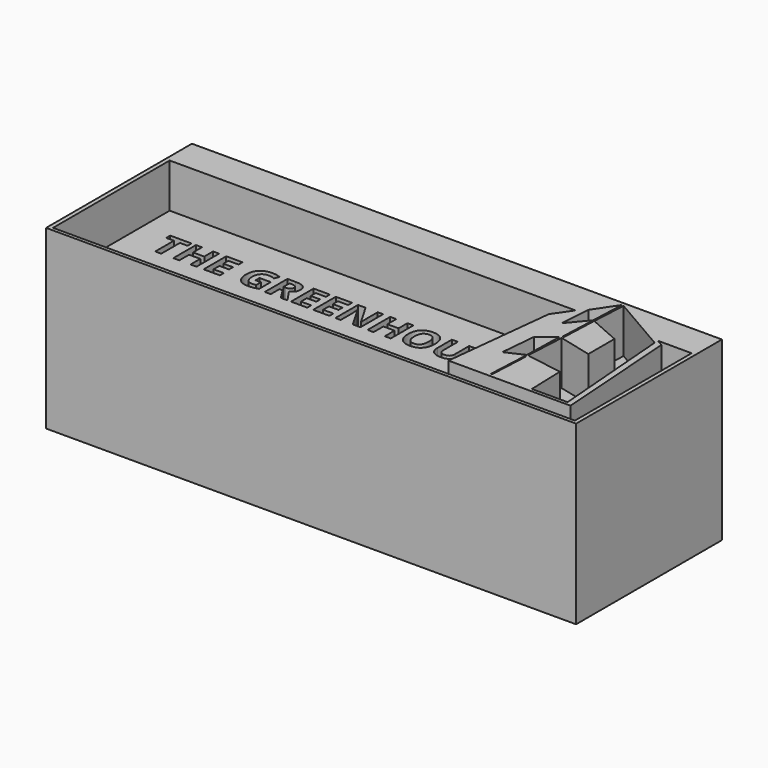
from build123d import *

# Parameters (mm, degrees)
F0_W           = 76.2
F0_H           = 26.2128
F0_TEXT_SIZE   = 6.6926038
F0_TEXT_SIZE_2 = 5.6983612304
F1_DEPTH       = 25.4
F2_DEPTH       = 6.35
F3_DEPTH       = 19.05
F4_DEPTH       = 6.35
F5_DEPTH       = 2.54


# Not quite as in the source:
# - Text() gives the source's letters only with a copy of the font that has no kerning and outlines rounded to 1/6400 em; it was checked with that copy


with BuildPart() as f1:
    # F0 (on Top) → F1 (new body)
    with BuildSketch(Plane.XY):
        with Locations((38.1, 13.1064)):
            Rectangle(F0_W, F0_H)
        Polygon((61.1613030252, 3.4926837004), (61.4434964955, 9.2476755381), (61.6211034358, 9.2712007463), (61.3373331726, 3.4840521403), align=None, mode=Mode.SUBTRACT)
        Polygon((0.6039433647, 0.4949280992), (0.6003574235, 21.4591026306), (58.9420162141, 21.4591026306), (57.1734681726, 18.863465637), (55.4423779249, 3.0197743326), (72.9824006557, 3.0197743326), (71.7260614038, 20.9190044552), (70.7809925079, 21.4808098972), (75.6342336535, 21.4808098972), (75.6342336535, 0.4949280992), align=None, mode=Mode.SUBTRACT)
        Polygon((58.8729605079, 8.4078907967), (59.333756566, 13.5073410347), (61.5762844682, 15.2632233005), (61.4434964955, 9.5933182165), align=None, mode=Mode.SUBTRACT)
        Polygon((72.1871778369, 3.4876975697), (67.0566137873, 3.4876975697), (66.889166832, 8.7119275704), (61.6209432483, 9.5933182165), (61.9224103407, 15.2632233005), (66.7000859976, 14.075903222), (66.7000859976, 18.7787953764), (62.214487733, 20.7565296441), (62.476977706, 25.6933644414), (70.8006359637, 20.868235606), align=None, mode=Mode.SUBTRACT)
        Polygon((61.7872286867, 15.5847425585), (61.9927414089, 20.6605475424), (62.2021403212, 20.6520692536), (61.996627599, 15.5762642697), align=None, mode=Mode.SUBTRACT)
        Polygon((62.1953939536, 25.7462535767), (61.996627599, 20.8370720795), (59.6932768822, 18.0755313486), (59.9989369512, 22.477010265), align=None, mode=Mode.SUBTRACT)
        Polygon((58.9420162141, 21.4591026306), (0.6003574235, 21.4591026306), (0.6039433647, 0.4949280992), (75.6342336535, 0.4949280992), (75.6342336535, 21.4808098972), (70.7809925079, 21.4808098972), (71.7260614038, 20.9190044552), (72.9824006557, 3.0197743326), (55.4423779249, 3.0197743326), (57.1734681726, 18.863465637), align=None)
        with BuildLine():
            Line((4.9192886227, 3.81), (4.9192886227, 8.5878916816))
            Line((4.9192886227, 8.5878916816), (6.4063015295, 8.5878916816))
            add(Edge.make_bspline(
                [(6.4063015295, 8.5878916816), (7.4227407316, 8.5878916816), (7.8818115235, 8.298750283)],
                knots=[0, 0, 0, 1, 1, 1], degree=2))
            add(Edge.make_bspline(
                [(7.8818115235, 8.298750283), (8.3408823154, 8.0096088845), (8.3408823154, 7.3790401202)],
                knots=[0, 0, 0, 1, 1, 1], degree=2))
            add(Edge.make_bspline(
                [(8.3408823154, 7.3790401202), (8.3408823154, 6.9502951893), (8.1401042014, 6.6757938615)],
                knots=[0, 0, 0, 1, 1, 1], degree=2))
            add(Edge.make_bspline(
                [(8.1401042014, 6.6757938615), (7.9393260874, 6.4012925338), (7.6057416167, 6.3458694086)],
                knots=[0, 0, 0, 1, 1, 1], degree=2))
            Line((7.6057416167, 6.3458694086), (7.6057416167, 6.3134521089))
            add(Edge.make_bspline(
                [(7.6057416167, 6.3134521089), (8.0595838119, 6.2120173326), (8.2608847856, 5.9343788468)],
                knots=[0, 0, 0, 1, 1, 1], degree=2))
            add(Edge.make_bspline(
                [(8.2608847856, 5.9343788468), (8.4621857593, 5.6567403611), (8.4621857593, 5.1955781305)],
                knots=[0, 0, 0, 1, 1, 1], degree=2))
            add(Edge.make_bspline(
                [(8.4621857593, 5.1955781305), (8.4621857593, 4.5420035406), (7.9895206159, 4.1760017703)],
                knots=[0, 0, 0, 1, 1, 1], degree=2))
            add(Edge.make_bspline(
                [(7.9895206159, 4.1760017703), (7.5168554725, 3.81), (6.7064229811, 3.81)],
                knots=[0, 0, 0, 1, 1, 1], degree=2))
            Line((6.7064229811, 3.81), (4.9192886227, 3.81))
        make_face(mode=Mode.SUBTRACT)
        with BuildLine():
            add(Edge.make_bspline(
                [(13.1689685255, 8.0289546924), (13.7524799193, 7.3947259104), (13.7524799193, 6.2057430165)],
                knots=[0, 0, 0, 1, 1, 1], degree=2))
            add(Edge.make_bspline(
                [(13.7524799193, 6.2057430165), (13.7524799193, 5.0188515614), (13.1642627884, 4.3814856214)],
                knots=[0, 0, 0, 1, 1, 1], degree=2))
            add(Edge.make_bspline(
                [(13.1642627884, 4.3814856214), (12.5760456576, 3.7441196813), (11.4780403467, 3.7441196813)],
                knots=[0, 0, 0, 1, 1, 1], degree=2))
            add(Edge.make_bspline(
                [(11.4780403467, 3.7441196813), (10.3800350357, 3.7441196813), (9.7918179049, 4.3814856214)],
                knots=[0, 0, 0, 1, 1, 1], degree=2))
            add(Edge.make_bspline(
                [(9.7918179049, 4.3814856214), (9.203600774, 5.0188515614), (9.203600774, 6.2120173326)],
                knots=[0, 0, 0, 1, 1, 1], degree=2))
            add(Edge.make_bspline(
                [(9.203600774, 6.2120173326), (9.203600774, 7.4051831038), (9.7933864839, 8.0341832891)],
                knots=[0, 0, 0, 1, 1, 1], degree=2))
            add(Edge.make_bspline(
                [(9.7933864839, 8.0341832891), (10.3831721937, 8.6631834743), (11.4843146627, 8.6631834743)],
                knots=[0, 0, 0, 1, 1, 1], degree=2))
            add(Edge.make_bspline(
                [(11.4843146627, 8.6631834743), (12.5854571317, 8.6631834743), (13.1689685255, 8.0289546924)],
                knots=[0, 0, 0, 1, 1, 1], degree=2))
        make_face(mode=Mode.SUBTRACT)
        Polygon((16.9910727269, 6.2182916487), (18.6056633936, 3.81), (17.4490977995, 3.81), (16.3374981371, 5.617003026), (15.226944194, 3.81), (14.1414875152, 3.81), (15.7267980403, 6.2737147739), (14.2429222915, 8.5878916816), (15.36079627, 8.5878916816), (16.3897841042, 6.8687290805), (17.3999489903, 8.5878916816), (18.4906342658, 8.5878916816), align=None, mode=Mode.SUBTRACT)
        with BuildLine():
            add(Edge.make_bspline(
                [(23.5079956771, 7.7183760473), (23.2371543671, 7.8130136479), (22.9757245312, 7.8130136479)],
                knots=[0, 0, 0, 1, 1, 1], degree=2))
            add(Edge.make_bspline(
                [(22.9757245312, 7.8130136479), (22.4037160501, 7.8130136479), (22.090000247, 7.3832229976)],
                knots=[0, 0, 0, 1, 1, 1], degree=2))
            add(Edge.make_bspline(
                [(22.090000247, 7.3832229976), (21.7762844439, 6.9534323473), (21.7762844439, 6.185874349)],
                knots=[0, 0, 0, 1, 1, 1], degree=2))
            add(Edge.make_bspline(
                [(21.7762844439, 6.185874349), (21.7762844439, 4.5880151917), (22.9757245312, 4.5880151917)],
                knots=[0, 0, 0, 1, 1, 1], degree=2))
            add(Edge.make_bspline(
                [(22.9757245312, 4.5880151917), (23.4787155355, 4.5880151917), (24.1939875666, 4.8389878342)],
                knots=[0, 0, 0, 1, 1, 1], degree=2))
            Line((24.1939875666, 4.8389878342), (24.1939875666, 3.9898637271))
            add(Edge.make_bspline(
                [(24.1939875666, 3.9898637271), (23.6062932955, 3.7441196813), (22.8805640709, 3.7441196813)],
                knots=[0, 0, 0, 1, 1, 1], degree=2))
            add(Edge.make_bspline(
                [(22.8805640709, 3.7441196813), (21.8379818852, 3.7441196813), (21.2858420717, 4.3767798843)],
                knots=[0, 0, 0, 1, 1, 1], degree=2))
            add(Edge.make_bspline(
                [(21.2858420717, 4.3767798843), (20.7337022582, 5.0094400873), (20.7337022582, 6.1921486651)],
                knots=[0, 0, 0, 1, 1, 1], degree=2))
            add(Edge.make_bspline(
                [(20.7337022582, 6.1921486651), (20.7337022582, 6.9377465572), (21.0050664279, 7.4982521254)],
                knots=[0, 0, 0, 1, 1, 1], degree=2))
            add(Edge.make_bspline(
                [(21.0050664279, 7.4982521254), (21.2764305976, 8.0587576937), (21.7846501986, 8.3573105663)],
                knots=[0, 0, 0, 1, 1, 1], degree=2))
            add(Edge.make_bspline(
                [(21.7846501986, 8.3573105663), (22.2928697997, 8.6558634389), (22.9757245312, 8.6558634389)],
                knots=[0, 0, 0, 1, 1, 1], degree=2))
            add(Edge.make_bspline(
                [(22.9757245312, 8.6558634389), (23.6711278948, 8.6558634389), (24.3738512938, 8.3201875296)],
                knots=[0, 0, 0, 1, 1, 1], degree=2))
            Line((24.3738512938, 8.3201875296), (24.0475868585, 7.4961606867))
            add(Edge.make_bspline(
                [(24.0475868585, 7.4961606867), (23.7788369872, 7.6237384467), (23.5079956771, 7.7183760473)],
                knots=[0, 0, 0, 1, 1, 1], degree=2))
        make_face(mode=Mode.SUBTRACT)
        with BuildLine():
            add(Edge.make_bspline(
                [(28.9635134935, 8.0289546924), (29.5470248873, 7.3947259104), (29.5470248873, 6.2057430165)],
                knots=[0, 0, 0, 1, 1, 1], degree=2))
            add(Edge.make_bspline(
                [(29.5470248873, 6.2057430165), (29.5470248873, 5.0188515614), (28.9588077564, 4.3814856214)],
                knots=[0, 0, 0, 1, 1, 1], degree=2))
            add(Edge.make_bspline(
                [(28.9588077564, 4.3814856214), (28.3705906256, 3.7441196813), (27.2725853146, 3.7441196813)],
                knots=[0, 0, 0, 1, 1, 1], degree=2))
            add(Edge.make_bspline(
                [(27.2725853146, 3.7441196813), (26.1745800037, 3.7441196813), (25.5863628728, 4.3814856214)],
                knots=[0, 0, 0, 1, 1, 1], degree=2))
            add(Edge.make_bspline(
                [(25.5863628728, 4.3814856214), (24.998145742, 5.0188515614), (24.998145742, 6.2120173326)],
                knots=[0, 0, 0, 1, 1, 1], degree=2))
            add(Edge.make_bspline(
                [(24.998145742, 6.2120173326), (24.998145742, 7.4051831038), (25.5879314519, 8.0341832891)],
                knots=[0, 0, 0, 1, 1, 1], degree=2))
            add(Edge.make_bspline(
                [(25.5879314519, 8.0341832891), (26.1777171617, 8.6631834743), (27.2788596307, 8.6631834743)],
                knots=[0, 0, 0, 1, 1, 1], degree=2))
            add(Edge.make_bspline(
                [(27.2788596307, 8.6631834743), (28.3800020997, 8.6631834743), (28.9635134935, 8.0289546924)],
                knots=[0, 0, 0, 1, 1, 1], degree=2))
        make_face(mode=Mode.SUBTRACT)
        with BuildLine():
            Line((33.4883410939, 3.81), (32.5597423166, 3.81))
            Line((32.5597423166, 3.81), (31.4094510385, 7.557858128))
            Line((31.4094510385, 7.557858128), (31.3801708969, 7.557858128))
            add(Edge.make_bspline(
                [(31.3801708969, 7.557858128), (31.4429140575, 6.4148868853), (31.4429140575, 6.0321536055)],
                knots=[0, 0, 0, 1, 1, 1], degree=2))
            Line((31.4429140575, 6.0321536055), (31.4429140575, 3.81))
            Line((31.4429140575, 3.81), (30.5373211058, 3.81))
            Line((30.5373211058, 3.81), (30.5373211058, 8.5878916816))
            Line((30.5373211058, 8.5878916816), (31.9166249202, 8.5878916816))
            Line((31.9166249202, 8.5878916816), (33.0470475308, 4.9341482945))
            Line((33.0470475308, 4.9341482945), (33.0669161984, 4.9341482945))
            Line((33.0669161984, 4.9341482945), (34.2663562856, 8.5878916816))
            Line((34.2663562856, 8.5878916816), (35.6446143807, 8.5878916816))
            Line((35.6446143807, 8.5878916816), (35.6446143807, 3.81))
            Line((35.6446143807, 3.81), (34.7003298133, 3.81))
            Line((34.7003298133, 3.81), (34.7003298133, 6.0718909405))
            add(Edge.make_bspline(
                [(34.7003298133, 6.0718909405), (34.7003298133, 6.2318860001), (34.70555841, 6.4410298689)],
                knots=[0, 0, 0, 1, 1, 1], degree=2))
            add(Edge.make_bspline(
                [(34.70555841, 6.4410298689), (34.7107870067, 6.6501737376), (34.7494786225, 7.5515838119)],
                knots=[0, 0, 0, 1, 1, 1], degree=2))
            Line((34.7494786225, 7.5515838119), (34.7201984808, 7.5515838119))
            Line((34.7201984808, 7.5515838119), (33.4883410939, 3.81))
        make_face(mode=Mode.SUBTRACT)
        with BuildLine():
            add(Edge.make_bspline(
                [(39.6952082587, 8.2135241565), (40.1474818749, 7.8391566315), (40.1474818749, 7.0977416167)],
                knots=[0, 0, 0, 1, 1, 1], degree=2))
            add(Edge.make_bspline(
                [(40.1474818749, 7.0977416167), (40.1474818749, 6.3260007411), (39.6654052574, 5.9176473373)],
                knots=[0, 0, 0, 1, 1, 1], degree=2))
            add(Edge.make_bspline(
                [(39.6654052574, 5.9176473373), (39.1833286399, 5.5092939336), (38.2944671978, 5.5092939336)],
                knots=[0, 0, 0, 1, 1, 1], degree=2))
            Line((38.2944671978, 5.5092939336), (37.8604936701, 5.5092939336))
            Line((37.8604936701, 5.5092939336), (37.8604936701, 3.81))
            Line((37.8604936701, 3.81), (36.847191626, 3.81))
            Line((36.847191626, 3.81), (36.847191626, 8.5878916816))
            Line((36.847191626, 8.5878916816), (38.3728961485, 8.5878916816))
            add(Edge.make_bspline(
                [(38.3728961485, 8.5878916816), (39.2429346425, 8.5878916816), (39.6952082587, 8.2135241565)],
                knots=[0, 0, 0, 1, 1, 1], degree=2))
        make_face(mode=Mode.SUBTRACT)
        Polygon((45.0665456679, 3.81), (43.974814673, 3.81), (43.6286815702, 4.947742646), (41.8865131435, 4.947742646), (41.5403800408, 3.81), (40.4486490459, 3.81), (42.1353943474, 8.6077603491), (43.3735260504, 8.6077603491), align=None, mode=Mode.SUBTRACT)
        with BuildLine():
            Line((49.9061347908, 8.5878916816), (49.9061347908, 3.81))
            Line((49.9061347908, 3.81), (48.6188542786, 3.81))
            Line((48.6188542786, 3.81), (46.5399642232, 7.424006052))
            Line((46.5399642232, 7.424006052), (46.5106840816, 7.424006052))
            add(Edge.make_bspline(
                [(46.5106840816, 7.424006052), (46.5734272422, 6.4671728525), (46.5734272422, 6.0582965891)],
                knots=[0, 0, 0, 1, 1, 1], degree=2))
            Line((46.5734272422, 6.0582965891), (46.5734272422, 3.81))
            Line((46.5734272422, 3.81), (45.6678342905, 3.81))
            Line((45.6678342905, 3.81), (45.6678342905, 8.5878916816))
            Line((45.6678342905, 8.5878916816), (46.9457033286, 8.5878916816))
            Line((46.9457033286, 8.5878916816), (49.0204105066, 5.0094400873))
            Line((49.0204105066, 5.0094400873), (49.0434163322, 5.0094400873))
            add(Edge.make_bspline(
                [(49.0434163322, 5.0094400873), (48.994267523, 5.9411760226), (48.994267523, 6.3260007411)],
                knots=[0, 0, 0, 1, 1, 1], degree=2))
            Line((48.994267523, 6.3260007411), (48.994267523, 8.5878916816))
            Line((48.994267523, 8.5878916816), (49.9061347908, 8.5878916816))
        make_face(mode=Mode.SUBTRACT)
        Polygon((51.6054287243, 8.5878916816), (52.5957249429, 6.620893596), (53.5922954775, 8.5878916816), (54.6840264723, 8.5878916816), (53.0987159472, 5.6692889932), (53.0987159472, 3.81), (52.0927339385, 3.81), (52.0927339385, 5.6368716935), (50.5074234134, 8.5878916816), align=None, mode=Mode.SUBTRACT)
        Polygon((6.399682587, 16.0504583297), (6.399682587, 12.7), (5.5369150819, 12.7), (5.5369150819, 16.0504583297), (4.4319672246, 16.0504583297), (4.4319672246, 16.7680956971), (7.5037400754, 16.7680956971), (7.5037400754, 16.0504583297), align=None, mode=Mode.SUBTRACT)
        Polygon((11.4632107615, 16.7680956971), (11.4632107615, 12.7), (10.6031143633, 12.7), (10.6031143633, 14.4558075541), (8.9924369468, 14.4558075541), (8.9924369468, 12.7), (8.1296694418, 12.7), (8.1296694418, 16.7680956971), (8.9924369468, 16.7680956971), (8.9924369468, 15.1734449216), (10.6031143633, 15.1734449216), (10.6031143633, 16.7680956971), align=None, mode=Mode.SUBTRACT)
        Polygon((14.832366839, 13.4122951538), (14.832366839, 12.7), (12.489806152, 12.7), (12.489806152, 16.7680956971), (14.832366839, 16.7680956971), (14.832366839, 16.061142757), (13.352573657, 16.061142757), (13.352573657, 15.1681027079), (14.7299744107, 15.1681027079), (14.7299744107, 14.4611497678), (13.352573657, 14.4611497678), (13.352573657, 13.4122951538), align=None, mode=Mode.SUBTRACT)
        with BuildLine():
            Line((18.7054717378, 14.2661589694), (18.7054717378, 14.9846867058))
            Line((18.7054717378, 14.9846867058), (20.3197106301, 14.9846867058))
            Line((20.3197106301, 14.9846867058), (20.3197106301, 12.8754026816))
            add(Edge.make_bspline(
                [(20.3197106301, 12.8754026816), (19.9270579266, 12.7471895539), (19.580704408, 12.6955481553)],
                knots=[0, 0, 0, 1, 1, 1], degree=2))
            add(Edge.make_bspline(
                [(19.580704408, 12.6955481553), (19.2343508895, 12.6439067566), (18.8728610989, 12.6439067566)],
                knots=[0, 0, 0, 1, 1, 1], degree=2))
            add(Edge.make_bspline(
                [(18.8728610989, 12.6439067566), (17.9522196127, 12.6439067566), (17.4665233547, 13.1852510735)],
                knots=[0, 0, 0, 1, 1, 1], degree=2))
            add(Edge.make_bspline(
                [(17.4665233547, 13.1852510735), (16.9808270967, 13.7265953904), (16.9808270967, 14.7398352467)],
                knots=[0, 0, 0, 1, 1, 1], degree=2))
            add(Edge.make_bspline(
                [(16.9808270967, 14.7398352467), (16.9808270967, 15.7245832968), (17.5444306371, 16.2752764876)],
                knots=[0, 0, 0, 1, 1, 1], degree=2))
            add(Edge.make_bspline(
                [(17.5444306371, 16.2752764876), (18.1080341775, 16.8259696784), (19.1061377618, 16.8259696784)],
                knots=[0, 0, 0, 1, 1, 1], degree=2))
            add(Edge.make_bspline(
                [(19.1061377618, 16.8259696784), (19.7329574972, 16.8259696784), (20.3143684164, 16.5757760056)],
                knots=[0, 0, 0, 1, 1, 1], degree=2))
            Line((20.3143684164, 16.5757760056), (20.027669617, 15.8857400754))
            add(Edge.make_bspline(
                [(20.027669617, 15.8857400754), (19.5824851459, 16.1083323109), (19.1007955482, 16.1083323109)],
                knots=[0, 0, 0, 1, 1, 1], degree=2))
            add(Edge.make_bspline(
                [(19.1007955482, 16.1083323109), (18.5416438524, 16.1083323109), (18.2050843923, 15.7325966173)],
                knots=[0, 0, 0, 1, 1, 1], degree=2))
            add(Edge.make_bspline(
                [(18.2050843923, 15.7325966173), (17.8685249321, 15.3568609237), (17.8685249321, 14.7229182368)],
                knots=[0, 0, 0, 1, 1, 1], degree=2))
            add(Edge.make_bspline(
                [(17.8685249321, 14.7229182368), (17.8685249321, 14.0604837438), (18.139642275, 13.7114591184)],
                knots=[0, 0, 0, 1, 1, 1], degree=2))
            add(Edge.make_bspline(
                [(18.139642275, 13.7114591184), (18.4107596179, 13.362434493), (18.9280639734, 13.362434493)],
                knots=[0, 0, 0, 1, 1, 1], degree=2))
            add(Edge.make_bspline(
                [(18.9280639734, 13.362434493), (19.1987361318, 13.362434493), (19.4765312418, 13.4176373675)],
                knots=[0, 0, 0, 1, 1, 1], degree=2))
            Line((19.4765312418, 13.4176373675), (19.4765312418, 14.2661589694))
            Line((19.4765312418, 14.2661589694), (18.7054717378, 14.2661589694))
        make_face(mode=Mode.SUBTRACT)
        with BuildLine():
            Line((22.6088491806, 14.2608167558), (22.1503091754, 14.2608167558))
            Line((22.1503091754, 14.2608167558), (22.1503091754, 12.7))
            Line((22.1503091754, 12.7), (21.2875416703, 12.7))
            Line((21.2875416703, 12.7), (21.2875416703, 16.7680956971))
            Line((21.2875416703, 16.7680956971), (22.4726227325, 16.7680956971))
            add(Edge.make_bspline(
                [(22.4726227325, 16.7680956971), (23.3024465866, 16.7680956971), (23.6999963193, 16.4662606257)],
                knots=[0, 0, 0, 1, 1, 1], degree=2))
            add(Edge.make_bspline(
                [(23.6999963193, 16.4662606257), (24.0975460521, 16.1644255543), (24.0975460521, 15.5491806152)],
                knots=[0, 0, 0, 1, 1, 1], degree=2))
            add(Edge.make_bspline(
                [(24.0975460521, 15.5491806152), (24.0975460521, 15.1903619315), (23.9003293313, 14.9107860836)],
                knots=[0, 0, 0, 1, 1, 1], degree=2))
            add(Edge.make_bspline(
                [(23.9003293313, 14.9107860836), (23.7031126106, 14.6312102357), (23.3407324511, 14.472724564)],
                knots=[0, 0, 0, 1, 1, 1], degree=2))
            add(Edge.make_bspline(
                [(23.3407324511, 14.472724564), (24.2595931995, 13.100666024), (24.5373883095, 12.7)],
                knots=[0, 0, 0, 1, 1, 1], degree=2))
            Line((24.5373883095, 12.7), (23.5802416966, 12.7))
            Line((23.5802416966, 12.7), (22.6088491806, 14.2608167558))
        make_face(mode=Mode.SUBTRACT)
        Polygon((27.3919111384, 13.4122951538), (27.3919111384, 12.7), (25.0493504513, 12.7), (25.0493504513, 16.7680956971), (27.3919111384, 16.7680956971), (27.3919111384, 16.061142757), (25.9121179564, 16.061142757), (25.9121179564, 15.1681027079), (27.28951871, 15.1681027079), (27.28951871, 14.4611497678), (25.9121179564, 14.4611497678), (25.9121179564, 13.4122951538), align=None, mode=Mode.SUBTRACT)
        Polygon((30.5829934274, 13.4122951538), (30.5829934274, 12.7), (28.2404327403, 12.7), (28.2404327403, 16.7680956971), (30.5829934274, 16.7680956971), (30.5829934274, 16.061142757), (29.1032002454, 16.061142757), (29.1032002454, 15.1681027079), (30.480600999, 15.1681027079), (30.480600999, 14.4611497678), (29.1032002454, 14.4611497678), (29.1032002454, 13.4122951538), align=None, mode=Mode.SUBTRACT)
        with BuildLine():
            Line((35.0401803523, 16.7680956971), (35.0401803523, 12.7))
            Line((35.0401803523, 12.7), (33.9441361844, 12.7))
            Line((33.9441361844, 12.7), (32.1740827272, 15.7771150644))
            Line((32.1740827272, 15.7771150644), (32.1491523968, 15.7771150644))
            add(Edge.make_bspline(
                [(32.1491523968, 15.7771150644), (32.2025745333, 14.9624274823), (32.2025745333, 14.6142932258)],
                knots=[0, 0, 0, 1, 1, 1], degree=2))
            Line((32.2025745333, 14.6142932258), (32.2025745333, 12.7))
            Line((32.2025745333, 12.7), (31.4315150294, 12.7))
            Line((31.4315150294, 12.7), (31.4315150294, 16.7680956971))
            Line((31.4315150294, 16.7680956971), (32.5195458768, 16.7680956971))
            Line((32.5195458768, 16.7680956971), (34.2860378582, 13.7212531768))
            Line((34.2860378582, 13.7212531768), (34.3056259749, 13.7212531768))
            add(Edge.make_bspline(
                [(34.3056259749, 13.7212531768), (34.2637786347, 14.5145719043), (34.2637786347, 14.8422276751)],
                knots=[0, 0, 0, 1, 1, 1], degree=2))
            Line((34.2637786347, 14.8422276751), (34.2637786347, 16.7680956971))
            Line((34.2637786347, 16.7680956971), (35.0401803523, 16.7680956971))
        make_face(mode=Mode.SUBTRACT)
        Polygon((39.3976459557, 16.7680956971), (39.3976459557, 12.7), (38.5375495574, 12.7), (38.5375495574, 14.4558075541), (36.9268721409, 14.4558075541), (36.9268721409, 12.7), (36.0641046359, 12.7), (36.0641046359, 16.7680956971), (36.9268721409, 16.7680956971), (36.9268721409, 15.1734449216), (38.5375495574, 15.1734449216), (38.5375495574, 16.7680956971), align=None, mode=Mode.SUBTRACT)
        with BuildLine():
            add(Edge.make_bspline(
                [(43.6197754798, 16.2921934975), (44.1166013496, 15.752184734), (44.1166013496, 14.7398352467)],
                knots=[0, 0, 0, 1, 1, 1], degree=2))
            add(Edge.make_bspline(
                [(44.1166013496, 14.7398352467), (44.1166013496, 13.7292664972), (43.6157688196, 13.1865866269)],
                knots=[0, 0, 0, 1, 1, 1], degree=2))
            add(Edge.make_bspline(
                [(43.6157688196, 13.1865866269), (43.1149362895, 12.6439067566), (42.1800489002, 12.6439067566)],
                knots=[0, 0, 0, 1, 1, 1], degree=2))
            add(Edge.make_bspline(
                [(42.1800489002, 12.6439067566), (41.2451615108, 12.6439067566), (40.7443289808, 13.1865866269)],
                knots=[0, 0, 0, 1, 1, 1], degree=2))
            add(Edge.make_bspline(
                [(40.7443289808, 13.1865866269), (40.2434964508, 13.7292664972), (40.2434964508, 14.7451774603)],
                knots=[0, 0, 0, 1, 1, 1], degree=2))
            add(Edge.make_bspline(
                [(40.2434964508, 14.7451774603), (40.2434964508, 15.7610884235), (40.7456645342, 16.2966453422)],
                knots=[0, 0, 0, 1, 1, 1], degree=2))
            add(Edge.make_bspline(
                [(40.7456645342, 16.2966453422), (41.2478326176, 16.832202261), (42.1853911138, 16.832202261)],
                knots=[0, 0, 0, 1, 1, 1], degree=2))
            add(Edge.make_bspline(
                [(42.1853911138, 16.832202261), (43.12294961, 16.832202261), (43.6197754798, 16.2921934975)],
                knots=[0, 0, 0, 1, 1, 1], degree=2))
        make_face(mode=Mode.SUBTRACT)
        with BuildLine():
            Line((47.4109664359, 16.7680956971), (48.2710628341, 16.7680956971))
            Line((48.2710628341, 16.7680956971), (48.2710628341, 14.1361651038))
            add(Edge.make_bspline(
                [(48.2710628341, 14.1361651038), (48.2710628341, 13.6847480501), (48.0693942687, 13.3455174831)],
                knots=[0, 0, 0, 1, 1, 1], degree=2))
            add(Edge.make_bspline(
                [(48.0693942687, 13.3455174831), (47.8677257033, 13.0062869161), (47.4862026115, 12.8250968364)],
                knots=[0, 0, 0, 1, 1, 1], degree=2))
            add(Edge.make_bspline(
                [(47.4862026115, 12.8250968364), (47.1046795198, 12.6439067566), (46.5847040575, 12.6439067566)],
                knots=[0, 0, 0, 1, 1, 1], degree=2))
            add(Edge.make_bspline(
                [(46.5847040575, 12.6439067566), (45.8002890194, 12.6439067566), (45.36623416, 13.0463535185)],
                knots=[0, 0, 0, 1, 1, 1], degree=2))
            add(Edge.make_bspline(
                [(45.36623416, 13.0463535185), (44.9321793007, 13.4488002804), (44.9321793007, 14.1468495312)],
                knots=[0, 0, 0, 1, 1, 1], degree=2))
            Line((44.9321793007, 14.1468495312), (44.9321793007, 16.7680956971))
            Line((44.9321793007, 16.7680956971), (45.7913853299, 16.7680956971))
            Line((45.7913853299, 16.7680956971), (45.7913853299, 14.2777337657))
            add(Edge.make_bspline(
                [(45.7913853299, 14.2777337657), (45.7913853299, 13.8076189642), (45.9805887302, 13.5876978354)],
                knots=[0, 0, 0, 1, 1, 1], degree=2))
            add(Edge.make_bspline(
                [(45.9805887302, 13.5876978354), (46.1697921304, 13.3677767067), (46.606963281, 13.3677767067)],
                knots=[0, 0, 0, 1, 1, 1], degree=2))
            add(Edge.make_bspline(
                [(46.606963281, 13.3677767067), (47.0298885286, 13.3677767067), (47.2204274823, 13.5890333888)],
                knots=[0, 0, 0, 1, 1, 1], degree=2))
            add(Edge.make_bspline(
                [(47.2204274823, 13.5890333888), (47.4109664359, 13.810290071), (47.4109664359, 14.2830759793)],
                knots=[0, 0, 0, 1, 1, 1], degree=2))
            Line((47.4109664359, 14.2830759793), (47.4109664359, 16.7680956971))
        make_face(mode=Mode.SUBTRACT)
        with BuildLine():
            add(Edge.make_bspline(
                [(51.4572480939, 14.5016615546), (51.6687107177, 14.2278731049), (51.6687107177, 13.8298781877)],
                knots=[0, 0, 0, 1, 1, 1], degree=2))
            add(Edge.make_bspline(
                [(51.6687107177, 13.8298781877), (51.6687107177, 13.2787398125), (51.272051354, 12.9613232845)],
                knots=[0, 0, 0, 1, 1, 1], degree=2))
            add(Edge.make_bspline(
                [(51.272051354, 12.9613232845), (50.8753919902, 12.6439067566), (50.169329419, 12.6439067566)],
                knots=[0, 0, 0, 1, 1, 1], degree=2))
            add(Edge.make_bspline(
                [(50.169329419, 12.6439067566), (49.5175793533, 12.6439067566), (49.0171920077, 12.8896485847)],
                knots=[0, 0, 0, 1, 1, 1], degree=2))
            Line((49.0171920077, 12.8896485847), (49.0171920077, 13.6909806327))
            add(Edge.make_bspline(
                [(49.0171920077, 13.6909806327), (49.428542459, 13.5066742617), (49.713905705, 13.4318832705)],
                knots=[0, 0, 0, 1, 1, 1], degree=2))
            add(Edge.make_bspline(
                [(49.713905705, 13.4318832705), (49.999268951, 13.3570922794), (50.2361070897, 13.3570922794)],
                knots=[0, 0, 0, 1, 1, 1], degree=2))
            add(Edge.make_bspline(
                [(50.2361070897, 13.3570922794), (50.5192444133, 13.3570922794), (50.6710523179, 13.4652721059)],
                knots=[0, 0, 0, 1, 1, 1], degree=2))
            add(Edge.make_bspline(
                [(50.6710523179, 13.4652721059), (50.8228602226, 13.5734519323), (50.8228602226, 13.7880308474)],
                knots=[0, 0, 0, 1, 1, 1], degree=2))
            add(Edge.make_bspline(
                [(50.8228602226, 13.7880308474), (50.8228602226, 13.9073402857), (50.7560825519, 14.0008290246)],
                knots=[0, 0, 0, 1, 1, 1], degree=2))
            add(Edge.make_bspline(
                [(50.7560825519, 14.0008290246), (50.6893048813, 14.0943177636), (50.5597562002, 14.1802383665)],
                knots=[0, 0, 0, 1, 1, 1], degree=2))
            add(Edge.make_bspline(
                [(50.5597562002, 14.1802383665), (50.4302075191, 14.2661589694), (50.0322126019, 14.4558075541)],
                knots=[0, 0, 0, 1, 1, 1], degree=2))
            add(Edge.make_bspline(
                [(50.0322126019, 14.4558075541), (49.660038384, 14.6312102357), (49.4735060906, 14.7923670143)],
                knots=[0, 0, 0, 1, 1, 1], degree=2))
            add(Edge.make_bspline(
                [(49.4735060906, 14.7923670143), (49.2869737972, 14.9535237928), (49.1756776794, 15.1681027079)],
                knots=[0, 0, 0, 1, 1, 1], degree=2))
            add(Edge.make_bspline(
                [(49.1756776794, 15.1681027079), (49.0643815617, 15.382681623), (49.0643815617, 15.6684900535)],
                knots=[0, 0, 0, 1, 1, 1], degree=2))
            add(Edge.make_bspline(
                [(49.0643815617, 15.6684900535), (49.0643815617, 16.2089440014), (49.4303231969, 16.5174568399)],
                knots=[0, 0, 0, 1, 1, 1], degree=2))
            add(Edge.make_bspline(
                [(49.4303231969, 16.5174568399), (49.7962648322, 16.8259696784), (50.4417823153, 16.8259696784)],
                knots=[0, 0, 0, 1, 1, 1], degree=2))
            add(Edge.make_bspline(
                [(50.4417823153, 16.8259696784), (50.7587536588, 16.8259696784), (51.0467880116, 16.7511786872)],
                knots=[0, 0, 0, 1, 1, 1], degree=2))
            add(Edge.make_bspline(
                [(51.0467880116, 16.7511786872), (51.3348223644, 16.6763876961), (51.649122601, 16.5401612479)],
                knots=[0, 0, 0, 1, 1, 1], degree=2))
            Line((51.649122601, 16.5401612479), (51.371327491, 15.8688230655))
            add(Edge.make_bspline(
                [(51.371327491, 15.8688230655), (51.0454524582, 16.0023784068), (50.832654281, 16.0553553589)],
                knots=[0, 0, 0, 1, 1, 1], degree=2))
            add(Edge.make_bspline(
                [(50.832654281, 16.0553553589), (50.6198561038, 16.1083323109), (50.4141808781, 16.1083323109)],
                knots=[0, 0, 0, 1, 1, 1], degree=2))
            add(Edge.make_bspline(
                [(50.4141808781, 16.1083323109), (50.169329419, 16.1083323109), (50.0384451845, 15.9943650863)],
                knots=[0, 0, 0, 1, 1, 1], degree=2))
            add(Edge.make_bspline(
                [(50.0384451845, 15.9943650863), (49.90756095, 15.8803978617), (49.90756095, 15.6969818596)],
                knots=[0, 0, 0, 1, 1, 1], degree=2))
            add(Edge.make_bspline(
                [(49.90756095, 15.6969818596), (49.90756095, 15.583014635), (49.960537902, 15.497984401)],
                knots=[0, 0, 0, 1, 1, 1], degree=2))
            add(Edge.make_bspline(
                [(49.960537902, 15.497984401), (50.0135148541, 15.412954167), (50.1288176321, 15.3337113312)],
                knots=[0, 0, 0, 1, 1, 1], degree=2))
            add(Edge.make_bspline(
                [(50.1288176321, 15.3337113312), (50.2441204101, 15.2544684953), (50.6750589782, 15.0487932697)],
                knots=[0, 0, 0, 1, 1, 1], degree=2))
            add(Edge.make_bspline(
                [(50.6750589782, 15.0487932697), (51.2457854702, 14.7754500044), (51.4572480939, 14.5016615546)],
                knots=[0, 0, 0, 1, 1, 1], degree=2))
        make_face(mode=Mode.SUBTRACT)
        Polygon((54.748496889, 13.4122951538), (54.748496889, 12.7), (52.4059362019, 12.7), (52.4059362019, 16.7680956971), (54.748496889, 16.7680956971), (54.748496889, 16.061142757), (53.2687037069, 16.061142757), (53.2687037069, 15.1681027079), (54.6461044606, 15.1681027079), (54.6461044606, 14.4611497678), (53.2687037069, 14.4611497678), (53.2687037069, 13.4122951538), align=None, mode=Mode.SUBTRACT)
        Polygon((66.889166832, 8.7119275704), (67.0566137873, 3.4876975697), (72.1871778369, 3.4876975697), (70.8006359637, 20.868235606), (62.476977706, 25.6933644414), (62.214487733, 20.7565296441), (66.7000859976, 18.7787953764), (66.7000859976, 14.075903222), (61.9224103407, 15.2632233005), (61.6209432483, 9.5933182165), align=None)
        Polygon((61.5762844682, 15.2632233005), (59.333756566, 13.5073410347), (58.8729605079, 8.4078907967), (61.4434964955, 9.5933182165), align=None)
        Polygon((59.6932768822, 18.0755313486), (61.996627599, 20.8370720795), (62.1953939536, 25.7462535767), (59.9989369512, 22.477010265), align=None)
        with Locations((4.318, 3.81)):
            Text('BOX COMPANY', F0_TEXT_SIZE, font='Open Sans', font_style=FontStyle.BOLD, text_align=(TextAlign.LEFT, TextAlign.BOTTOM))
        with BuildLine():
            add(Edge.make_bspline(
                [(26.3675152226, 7.4125031392), (26.0605965952, 7.0057183145), (26.0605965952, 6.2057430165)],
                knots=[0, 0, 0, 1, 1, 1], degree=2))
            add(Edge.make_bspline(
                [(26.0605965952, 6.2057430165), (26.0605965952, 5.4047219992), (26.3643780646, 4.9995057535)],
                knots=[0, 0, 0, 1, 1, 1], degree=2))
            add(Edge.make_bspline(
                [(26.3643780646, 4.9995057535), (26.668159534, 4.5942895078), (27.2725853146, 4.5942895078)],
                knots=[0, 0, 0, 1, 1, 1], degree=2))
            add(Edge.make_bspline(
                [(27.2725853146, 4.5942895078), (28.484574034, 4.5942895078), (28.484574034, 6.2057430165)],
                knots=[0, 0, 0, 1, 1, 1], degree=2))
            add(Edge.make_bspline(
                [(28.484574034, 6.2057430165), (28.484574034, 7.8192879639), (27.2788596307, 7.8192879639)],
                knots=[0, 0, 0, 1, 1, 1], degree=2))
            add(Edge.make_bspline(
                [(27.2788596307, 7.8192879639), (26.67443385, 7.8192879639), (26.3675152226, 7.4125031392)],
                knots=[0, 0, 0, 1, 1, 1], degree=2))
        make_face()
        with BuildLine():
            add(Edge.make_bspline(
                [(10.5729702546, 7.4125031392), (10.2660516272, 7.0057183145), (10.2660516272, 6.2057430165)],
                knots=[0, 0, 0, 1, 1, 1], degree=2))
            add(Edge.make_bspline(
                [(10.2660516272, 6.2057430165), (10.2660516272, 5.4047219992), (10.5698330966, 4.9995057535)],
                knots=[0, 0, 0, 1, 1, 1], degree=2))
            add(Edge.make_bspline(
                [(10.5698330966, 4.9995057535), (10.873614566, 4.5942895078), (11.4780403467, 4.5942895078)],
                knots=[0, 0, 0, 1, 1, 1], degree=2))
            add(Edge.make_bspline(
                [(11.4780403467, 4.5942895078), (12.6900290661, 4.5942895078), (12.6900290661, 6.2057430165)],
                knots=[0, 0, 0, 1, 1, 1], degree=2))
            add(Edge.make_bspline(
                [(12.6900290661, 6.2057430165), (12.6900290661, 7.8192879639), (11.4843146627, 7.8192879639)],
                knots=[0, 0, 0, 1, 1, 1], degree=2))
            add(Edge.make_bspline(
                [(11.4843146627, 7.8192879639), (10.879888882, 7.8192879639), (10.5729702546, 7.4125031392)],
                knots=[0, 0, 0, 1, 1, 1], degree=2))
        make_face()
        with Locations((4.318, 12.7)):
            Text('THE GREENHOUSE', F0_TEXT_SIZE_2, font='Open Sans', font_style=FontStyle.BOLD, text_align=(TextAlign.LEFT, TextAlign.BOTTOM))
        with BuildLine():
            add(Edge.make_bspline(
                [(41.4094345807, 15.767321006), (41.1481112961, 15.4209674875), (41.1481112961, 14.7398352467)],
                knots=[0, 0, 0, 1, 1, 1], degree=2))
            add(Edge.make_bspline(
                [(41.1481112961, 14.7398352467), (41.1481112961, 14.0578126369), (41.4067634738, 13.7127946718)],
                knots=[0, 0, 0, 1, 1, 1], degree=2))
            add(Edge.make_bspline(
                [(41.4067634738, 13.7127946718), (41.6654156516, 13.3677767067), (42.1800489002, 13.3677767067)],
                knots=[0, 0, 0, 1, 1, 1], degree=2))
            add(Edge.make_bspline(
                [(42.1800489002, 13.3677767067), (43.2119865043, 13.3677767067), (43.2119865043, 14.7398352467)],
                knots=[0, 0, 0, 1, 1, 1], degree=2))
            add(Edge.make_bspline(
                [(43.2119865043, 14.7398352467), (43.2119865043, 16.1136745246), (42.1853911138, 16.1136745246)],
                knots=[0, 0, 0, 1, 1, 1], degree=2))
            add(Edge.make_bspline(
                [(42.1853911138, 16.1136745246), (41.6707578652, 16.1136745246), (41.4094345807, 15.767321006)],
                knots=[0, 0, 0, 1, 1, 1], degree=2))
        make_face()
        with BuildLine():
            Line((6.560022273, 5.8920272134), (5.9325906667, 5.8920272134))
            Line((5.9325906667, 5.8920272134), (5.9325906667, 4.646575475))
            Line((5.9325906667, 4.646575475), (6.5924395727, 4.646575475))
            add(Edge.make_bspline(
                [(6.5924395727, 4.646575475), (7.0107273102, 4.646575475), (7.2099368451, 4.8065705346)],
                knots=[0, 0, 0, 1, 1, 1], degree=2))
            add(Edge.make_bspline(
                [(7.2099368451, 4.8065705346), (7.4091463801, 4.9665655942), (7.4091463801, 5.2970129068)],
                knots=[0, 0, 0, 1, 1, 1], degree=2))
            add(Edge.make_bspline(
                [(7.4091463801, 5.2970129068), (7.4091463801, 5.8920272134), (6.560022273, 5.8920272134)],
                knots=[0, 0, 0, 1, 1, 1], degree=2))
        make_face()
        with BuildLine():
            Line((37.8604936701, 7.7575905227), (37.8604936701, 6.3395950925))
            Line((37.8604936701, 6.3395950925), (38.1940781408, 6.3395950925))
            add(Edge.make_bspline(
                [(38.1940781408, 6.3395950925), (38.6604689681, 6.3395950925), (38.8926186624, 6.5241645567)],
                knots=[0, 0, 0, 1, 1, 1], degree=2))
            add(Edge.make_bspline(
                [(38.8926186624, 6.5241645567), (39.1247683567, 6.7087340209), (39.1247683567, 7.0611414397)],
                knots=[0, 0, 0, 1, 1, 1], degree=2))
            add(Edge.make_bspline(
                [(39.1247683567, 7.0611414397), (39.1247683567, 7.4177317359), (38.9302645588, 7.5876611293)],
                knots=[0, 0, 0, 1, 1, 1], degree=2))
            add(Edge.make_bspline(
                [(38.9302645588, 7.5876611293), (38.7357607608, 7.7575905227), (38.3206101814, 7.7575905227)],
                knots=[0, 0, 0, 1, 1, 1], degree=2))
            Line((38.3206101814, 7.7575905227), (37.8604936701, 7.7575905227))
        make_face()
        with BuildLine():
            Line((5.9325906667, 7.7575905227), (5.9325906667, 6.6951396694))
            Line((5.9325906667, 6.6951396694), (6.5202849379, 6.6951396694))
            add(Edge.make_bspline(
                [(6.5202849379, 6.6951396694), (6.9322983594, 6.6951396694), (7.1168678235, 6.8227174293)],
                knots=[0, 0, 0, 1, 1, 1], degree=2))
            add(Edge.make_bspline(
                [(7.1168678235, 6.8227174293), (7.3014372877, 6.9502951893), (7.3014372877, 7.2441423249)],
                knots=[0, 0, 0, 1, 1, 1], degree=2))
            add(Edge.make_bspline(
                [(7.3014372877, 7.2441423249), (7.3014372877, 7.5191665123), (7.1006591737, 7.6383785175)],
                knots=[0, 0, 0, 1, 1, 1], degree=2))
            add(Edge.make_bspline(
                [(7.1006591737, 7.6383785175), (6.8998810597, 7.7575905227), (6.4648618127, 7.7575905227)],
                knots=[0, 0, 0, 1, 1, 1], degree=2))
            Line((6.4648618127, 7.7575905227), (5.9325906667, 7.7575905227))
        make_face()
        with BuildLine():
            Line((42.1416686634, 5.7968667531), (43.3860746825, 5.7968667531))
            add(Edge.make_bspline(
                [(43.3860746825, 5.7968667531), (42.9060895037, 7.3424399432), (42.8454377818, 7.5453094959)],
                knots=[0, 0, 0, 1, 1, 1], degree=2))
            add(Edge.make_bspline(
                [(42.8454377818, 7.5453094959), (42.7847860598, 7.7481790486), (42.7586430762, 7.8652996151)],
                knots=[0, 0, 0, 1, 1, 1], degree=2))
            add(Edge.make_bspline(
                [(42.7586430762, 7.8652996151), (42.6509339838, 7.4470118776), (42.1416686634, 5.7968667531)],
                knots=[0, 0, 0, 1, 1, 1], degree=2))
        make_face()
        Polygon((62.2021403212, 20.6520692536), (61.9927414089, 20.6605475424), (61.7872286867, 15.5847425585), (61.996627599, 15.5762642697), align=None)
        with BuildLine():
            Line((22.1503091754, 16.061142757), (22.1503091754, 14.9624274823))
            Line((22.1503091754, 14.9624274823), (22.4281042853, 14.9624274823))
            add(Edge.make_bspline(
                [(22.4281042853, 14.9624274823), (22.8376739988, 14.9624274823), (23.0322196127, 15.0986539304)],
                knots=[0, 0, 0, 1, 1, 1], degree=2))
            add(Edge.make_bspline(
                [(23.0322196127, 15.0986539304), (23.2267652265, 15.2348803786), (23.2267652265, 15.5269213916)],
                knots=[0, 0, 0, 1, 1, 1], degree=2))
            add(Edge.make_bspline(
                [(23.2267652265, 15.5269213916), (23.2267652265, 15.8162912979), (23.0277677679, 15.9387170274)],
                knots=[0, 0, 0, 1, 1, 1], degree=2))
            add(Edge.make_bspline(
                [(23.0277677679, 15.9387170274), (22.8287703094, 16.061142757), (22.4120776444, 16.061142757)],
                knots=[0, 0, 0, 1, 1, 1], degree=2))
            Line((22.4120776444, 16.061142757), (22.1503091754, 16.061142757))
        make_face()
        Polygon((61.6211034358, 9.2712007463), (61.4434964955, 9.2476755381), (61.1613030252, 3.4926837004), (61.3373331726, 3.4840521403), align=None)
    extrude(amount=-F1_DEPTH)

    # F0 (on Top) → F2 (cut)
    with BuildSketch(Plane.XY):
        Polygon((58.9420162141, 21.4591026306), (0.6003574235, 21.4591026306), (0.6039433647, 0.4949280992), (75.6342336535, 0.4949280992), (75.6342336535, 21.4808098972), (70.7809925079, 21.4808098972), (71.7260614038, 20.9190044552), (72.9824006557, 3.0197743326), (55.4423779249, 3.0197743326), (57.1734681726, 18.863465637), align=None)
        with BuildLine():
            Line((4.9192886227, 3.81), (4.9192886227, 8.5878916816))
            Line((4.9192886227, 8.5878916816), (6.4063015295, 8.5878916816))
            add(Edge.make_bspline(
                [(6.4063015295, 8.5878916816), (7.4227407316, 8.5878916816), (7.8818115235, 8.298750283)],
                knots=[0, 0, 0, 1, 1, 1], degree=2))
            add(Edge.make_bspline(
                [(7.8818115235, 8.298750283), (8.3408823154, 8.0096088845), (8.3408823154, 7.3790401202)],
                knots=[0, 0, 0, 1, 1, 1], degree=2))
            add(Edge.make_bspline(
                [(8.3408823154, 7.3790401202), (8.3408823154, 6.9502951893), (8.1401042014, 6.6757938615)],
                knots=[0, 0, 0, 1, 1, 1], degree=2))
            add(Edge.make_bspline(
                [(8.1401042014, 6.6757938615), (7.9393260874, 6.4012925338), (7.6057416167, 6.3458694086)],
                knots=[0, 0, 0, 1, 1, 1], degree=2))
            Line((7.6057416167, 6.3458694086), (7.6057416167, 6.3134521089))
            add(Edge.make_bspline(
                [(7.6057416167, 6.3134521089), (8.0595838119, 6.2120173326), (8.2608847856, 5.9343788468)],
                knots=[0, 0, 0, 1, 1, 1], degree=2))
            add(Edge.make_bspline(
                [(8.2608847856, 5.9343788468), (8.4621857593, 5.6567403611), (8.4621857593, 5.1955781305)],
                knots=[0, 0, 0, 1, 1, 1], degree=2))
            add(Edge.make_bspline(
                [(8.4621857593, 5.1955781305), (8.4621857593, 4.5420035406), (7.9895206159, 4.1760017703)],
                knots=[0, 0, 0, 1, 1, 1], degree=2))
            add(Edge.make_bspline(
                [(7.9895206159, 4.1760017703), (7.5168554725, 3.81), (6.7064229811, 3.81)],
                knots=[0, 0, 0, 1, 1, 1], degree=2))
            Line((6.7064229811, 3.81), (4.9192886227, 3.81))
        make_face(mode=Mode.SUBTRACT)
        with BuildLine():
            add(Edge.make_bspline(
                [(13.1689685255, 8.0289546924), (13.7524799193, 7.3947259104), (13.7524799193, 6.2057430165)],
                knots=[0, 0, 0, 1, 1, 1], degree=2))
            add(Edge.make_bspline(
                [(13.7524799193, 6.2057430165), (13.7524799193, 5.0188515614), (13.1642627884, 4.3814856214)],
                knots=[0, 0, 0, 1, 1, 1], degree=2))
            add(Edge.make_bspline(
                [(13.1642627884, 4.3814856214), (12.5760456576, 3.7441196813), (11.4780403467, 3.7441196813)],
                knots=[0, 0, 0, 1, 1, 1], degree=2))
            add(Edge.make_bspline(
                [(11.4780403467, 3.7441196813), (10.3800350357, 3.7441196813), (9.7918179049, 4.3814856214)],
                knots=[0, 0, 0, 1, 1, 1], degree=2))
            add(Edge.make_bspline(
                [(9.7918179049, 4.3814856214), (9.203600774, 5.0188515614), (9.203600774, 6.2120173326)],
                knots=[0, 0, 0, 1, 1, 1], degree=2))
            add(Edge.make_bspline(
                [(9.203600774, 6.2120173326), (9.203600774, 7.4051831038), (9.7933864839, 8.0341832891)],
                knots=[0, 0, 0, 1, 1, 1], degree=2))
            add(Edge.make_bspline(
                [(9.7933864839, 8.0341832891), (10.3831721937, 8.6631834743), (11.4843146627, 8.6631834743)],
                knots=[0, 0, 0, 1, 1, 1], degree=2))
            add(Edge.make_bspline(
                [(11.4843146627, 8.6631834743), (12.5854571317, 8.6631834743), (13.1689685255, 8.0289546924)],
                knots=[0, 0, 0, 1, 1, 1], degree=2))
        make_face(mode=Mode.SUBTRACT)
        Polygon((16.9910727269, 6.2182916487), (18.6056633936, 3.81), (17.4490977995, 3.81), (16.3374981371, 5.617003026), (15.226944194, 3.81), (14.1414875152, 3.81), (15.7267980403, 6.2737147739), (14.2429222915, 8.5878916816), (15.36079627, 8.5878916816), (16.3897841042, 6.8687290805), (17.3999489903, 8.5878916816), (18.4906342658, 8.5878916816), align=None, mode=Mode.SUBTRACT)
        with BuildLine():
            add(Edge.make_bspline(
                [(23.5079956771, 7.7183760473), (23.2371543671, 7.8130136479), (22.9757245312, 7.8130136479)],
                knots=[0, 0, 0, 1, 1, 1], degree=2))
            add(Edge.make_bspline(
                [(22.9757245312, 7.8130136479), (22.4037160501, 7.8130136479), (22.090000247, 7.3832229976)],
                knots=[0, 0, 0, 1, 1, 1], degree=2))
            add(Edge.make_bspline(
                [(22.090000247, 7.3832229976), (21.7762844439, 6.9534323473), (21.7762844439, 6.185874349)],
                knots=[0, 0, 0, 1, 1, 1], degree=2))
            add(Edge.make_bspline(
                [(21.7762844439, 6.185874349), (21.7762844439, 4.5880151917), (22.9757245312, 4.5880151917)],
                knots=[0, 0, 0, 1, 1, 1], degree=2))
            add(Edge.make_bspline(
                [(22.9757245312, 4.5880151917), (23.4787155355, 4.5880151917), (24.1939875666, 4.8389878342)],
                knots=[0, 0, 0, 1, 1, 1], degree=2))
            Line((24.1939875666, 4.8389878342), (24.1939875666, 3.9898637271))
            add(Edge.make_bspline(
                [(24.1939875666, 3.9898637271), (23.6062932955, 3.7441196813), (22.8805640709, 3.7441196813)],
                knots=[0, 0, 0, 1, 1, 1], degree=2))
            add(Edge.make_bspline(
                [(22.8805640709, 3.7441196813), (21.8379818852, 3.7441196813), (21.2858420717, 4.3767798843)],
                knots=[0, 0, 0, 1, 1, 1], degree=2))
            add(Edge.make_bspline(
                [(21.2858420717, 4.3767798843), (20.7337022582, 5.0094400873), (20.7337022582, 6.1921486651)],
                knots=[0, 0, 0, 1, 1, 1], degree=2))
            add(Edge.make_bspline(
                [(20.7337022582, 6.1921486651), (20.7337022582, 6.9377465572), (21.0050664279, 7.4982521254)],
                knots=[0, 0, 0, 1, 1, 1], degree=2))
            add(Edge.make_bspline(
                [(21.0050664279, 7.4982521254), (21.2764305976, 8.0587576937), (21.7846501986, 8.3573105663)],
                knots=[0, 0, 0, 1, 1, 1], degree=2))
            add(Edge.make_bspline(
                [(21.7846501986, 8.3573105663), (22.2928697997, 8.6558634389), (22.9757245312, 8.6558634389)],
                knots=[0, 0, 0, 1, 1, 1], degree=2))
            add(Edge.make_bspline(
                [(22.9757245312, 8.6558634389), (23.6711278948, 8.6558634389), (24.3738512938, 8.3201875296)],
                knots=[0, 0, 0, 1, 1, 1], degree=2))
            Line((24.3738512938, 8.3201875296), (24.0475868585, 7.4961606867))
            add(Edge.make_bspline(
                [(24.0475868585, 7.4961606867), (23.7788369872, 7.6237384467), (23.5079956771, 7.7183760473)],
                knots=[0, 0, 0, 1, 1, 1], degree=2))
        make_face(mode=Mode.SUBTRACT)
        with BuildLine():
            add(Edge.make_bspline(
                [(28.9635134935, 8.0289546924), (29.5470248873, 7.3947259104), (29.5470248873, 6.2057430165)],
                knots=[0, 0, 0, 1, 1, 1], degree=2))
            add(Edge.make_bspline(
                [(29.5470248873, 6.2057430165), (29.5470248873, 5.0188515614), (28.9588077564, 4.3814856214)],
                knots=[0, 0, 0, 1, 1, 1], degree=2))
            add(Edge.make_bspline(
                [(28.9588077564, 4.3814856214), (28.3705906256, 3.7441196813), (27.2725853146, 3.7441196813)],
                knots=[0, 0, 0, 1, 1, 1], degree=2))
            add(Edge.make_bspline(
                [(27.2725853146, 3.7441196813), (26.1745800037, 3.7441196813), (25.5863628728, 4.3814856214)],
                knots=[0, 0, 0, 1, 1, 1], degree=2))
            add(Edge.make_bspline(
                [(25.5863628728, 4.3814856214), (24.998145742, 5.0188515614), (24.998145742, 6.2120173326)],
                knots=[0, 0, 0, 1, 1, 1], degree=2))
            add(Edge.make_bspline(
                [(24.998145742, 6.2120173326), (24.998145742, 7.4051831038), (25.5879314519, 8.0341832891)],
                knots=[0, 0, 0, 1, 1, 1], degree=2))
            add(Edge.make_bspline(
                [(25.5879314519, 8.0341832891), (26.1777171617, 8.6631834743), (27.2788596307, 8.6631834743)],
                knots=[0, 0, 0, 1, 1, 1], degree=2))
            add(Edge.make_bspline(
                [(27.2788596307, 8.6631834743), (28.3800020997, 8.6631834743), (28.9635134935, 8.0289546924)],
                knots=[0, 0, 0, 1, 1, 1], degree=2))
        make_face(mode=Mode.SUBTRACT)
        with BuildLine():
            Line((33.4883410939, 3.81), (32.5597423166, 3.81))
            Line((32.5597423166, 3.81), (31.4094510385, 7.557858128))
            Line((31.4094510385, 7.557858128), (31.3801708969, 7.557858128))
            add(Edge.make_bspline(
                [(31.3801708969, 7.557858128), (31.4429140575, 6.4148868853), (31.4429140575, 6.0321536055)],
                knots=[0, 0, 0, 1, 1, 1], degree=2))
            Line((31.4429140575, 6.0321536055), (31.4429140575, 3.81))
            Line((31.4429140575, 3.81), (30.5373211058, 3.81))
            Line((30.5373211058, 3.81), (30.5373211058, 8.5878916816))
            Line((30.5373211058, 8.5878916816), (31.9166249202, 8.5878916816))
            Line((31.9166249202, 8.5878916816), (33.0470475308, 4.9341482945))
            Line((33.0470475308, 4.9341482945), (33.0669161984, 4.9341482945))
            Line((33.0669161984, 4.9341482945), (34.2663562856, 8.5878916816))
            Line((34.2663562856, 8.5878916816), (35.6446143807, 8.5878916816))
            Line((35.6446143807, 8.5878916816), (35.6446143807, 3.81))
            Line((35.6446143807, 3.81), (34.7003298133, 3.81))
            Line((34.7003298133, 3.81), (34.7003298133, 6.0718909405))
            add(Edge.make_bspline(
                [(34.7003298133, 6.0718909405), (34.7003298133, 6.2318860001), (34.70555841, 6.4410298689)],
                knots=[0, 0, 0, 1, 1, 1], degree=2))
            add(Edge.make_bspline(
                [(34.70555841, 6.4410298689), (34.7107870067, 6.6501737376), (34.7494786225, 7.5515838119)],
                knots=[0, 0, 0, 1, 1, 1], degree=2))
            Line((34.7494786225, 7.5515838119), (34.7201984808, 7.5515838119))
            Line((34.7201984808, 7.5515838119), (33.4883410939, 3.81))
        make_face(mode=Mode.SUBTRACT)
        with BuildLine():
            add(Edge.make_bspline(
                [(39.6952082587, 8.2135241565), (40.1474818749, 7.8391566315), (40.1474818749, 7.0977416167)],
                knots=[0, 0, 0, 1, 1, 1], degree=2))
            add(Edge.make_bspline(
                [(40.1474818749, 7.0977416167), (40.1474818749, 6.3260007411), (39.6654052574, 5.9176473373)],
                knots=[0, 0, 0, 1, 1, 1], degree=2))
            add(Edge.make_bspline(
                [(39.6654052574, 5.9176473373), (39.1833286399, 5.5092939336), (38.2944671978, 5.5092939336)],
                knots=[0, 0, 0, 1, 1, 1], degree=2))
            Line((38.2944671978, 5.5092939336), (37.8604936701, 5.5092939336))
            Line((37.8604936701, 5.5092939336), (37.8604936701, 3.81))
            Line((37.8604936701, 3.81), (36.847191626, 3.81))
            Line((36.847191626, 3.81), (36.847191626, 8.5878916816))
            Line((36.847191626, 8.5878916816), (38.3728961485, 8.5878916816))
            add(Edge.make_bspline(
                [(38.3728961485, 8.5878916816), (39.2429346425, 8.5878916816), (39.6952082587, 8.2135241565)],
                knots=[0, 0, 0, 1, 1, 1], degree=2))
        make_face(mode=Mode.SUBTRACT)
        Polygon((45.0665456679, 3.81), (43.974814673, 3.81), (43.6286815702, 4.947742646), (41.8865131435, 4.947742646), (41.5403800408, 3.81), (40.4486490459, 3.81), (42.1353943474, 8.6077603491), (43.3735260504, 8.6077603491), align=None, mode=Mode.SUBTRACT)
        with BuildLine():
            Line((49.9061347908, 8.5878916816), (49.9061347908, 3.81))
            Line((49.9061347908, 3.81), (48.6188542786, 3.81))
            Line((48.6188542786, 3.81), (46.5399642232, 7.424006052))
            Line((46.5399642232, 7.424006052), (46.5106840816, 7.424006052))
            add(Edge.make_bspline(
                [(46.5106840816, 7.424006052), (46.5734272422, 6.4671728525), (46.5734272422, 6.0582965891)],
                knots=[0, 0, 0, 1, 1, 1], degree=2))
            Line((46.5734272422, 6.0582965891), (46.5734272422, 3.81))
            Line((46.5734272422, 3.81), (45.6678342905, 3.81))
            Line((45.6678342905, 3.81), (45.6678342905, 8.5878916816))
            Line((45.6678342905, 8.5878916816), (46.9457033286, 8.5878916816))
            Line((46.9457033286, 8.5878916816), (49.0204105066, 5.0094400873))
            Line((49.0204105066, 5.0094400873), (49.0434163322, 5.0094400873))
            add(Edge.make_bspline(
                [(49.0434163322, 5.0094400873), (48.994267523, 5.9411760226), (48.994267523, 6.3260007411)],
                knots=[0, 0, 0, 1, 1, 1], degree=2))
            Line((48.994267523, 6.3260007411), (48.994267523, 8.5878916816))
            Line((48.994267523, 8.5878916816), (49.9061347908, 8.5878916816))
        make_face(mode=Mode.SUBTRACT)
        Polygon((51.6054287243, 8.5878916816), (52.5957249429, 6.620893596), (53.5922954775, 8.5878916816), (54.6840264723, 8.5878916816), (53.0987159472, 5.6692889932), (53.0987159472, 3.81), (52.0927339385, 3.81), (52.0927339385, 5.6368716935), (50.5074234134, 8.5878916816), align=None, mode=Mode.SUBTRACT)
        Polygon((6.399682587, 16.0504583297), (6.399682587, 12.7), (5.5369150819, 12.7), (5.5369150819, 16.0504583297), (4.4319672246, 16.0504583297), (4.4319672246, 16.7680956971), (7.5037400754, 16.7680956971), (7.5037400754, 16.0504583297), align=None, mode=Mode.SUBTRACT)
        Polygon((11.4632107615, 16.7680956971), (11.4632107615, 12.7), (10.6031143633, 12.7), (10.6031143633, 14.4558075541), (8.9924369468, 14.4558075541), (8.9924369468, 12.7), (8.1296694418, 12.7), (8.1296694418, 16.7680956971), (8.9924369468, 16.7680956971), (8.9924369468, 15.1734449216), (10.6031143633, 15.1734449216), (10.6031143633, 16.7680956971), align=None, mode=Mode.SUBTRACT)
        Polygon((14.832366839, 13.4122951538), (14.832366839, 12.7), (12.489806152, 12.7), (12.489806152, 16.7680956971), (14.832366839, 16.7680956971), (14.832366839, 16.061142757), (13.352573657, 16.061142757), (13.352573657, 15.1681027079), (14.7299744107, 15.1681027079), (14.7299744107, 14.4611497678), (13.352573657, 14.4611497678), (13.352573657, 13.4122951538), align=None, mode=Mode.SUBTRACT)
        with BuildLine():
            Line((18.7054717378, 14.2661589694), (18.7054717378, 14.9846867058))
            Line((18.7054717378, 14.9846867058), (20.3197106301, 14.9846867058))
            Line((20.3197106301, 14.9846867058), (20.3197106301, 12.8754026816))
            add(Edge.make_bspline(
                [(20.3197106301, 12.8754026816), (19.9270579266, 12.7471895539), (19.580704408, 12.6955481553)],
                knots=[0, 0, 0, 1, 1, 1], degree=2))
            add(Edge.make_bspline(
                [(19.580704408, 12.6955481553), (19.2343508895, 12.6439067566), (18.8728610989, 12.6439067566)],
                knots=[0, 0, 0, 1, 1, 1], degree=2))
            add(Edge.make_bspline(
                [(18.8728610989, 12.6439067566), (17.9522196127, 12.6439067566), (17.4665233547, 13.1852510735)],
                knots=[0, 0, 0, 1, 1, 1], degree=2))
            add(Edge.make_bspline(
                [(17.4665233547, 13.1852510735), (16.9808270967, 13.7265953904), (16.9808270967, 14.7398352467)],
                knots=[0, 0, 0, 1, 1, 1], degree=2))
            add(Edge.make_bspline(
                [(16.9808270967, 14.7398352467), (16.9808270967, 15.7245832968), (17.5444306371, 16.2752764876)],
                knots=[0, 0, 0, 1, 1, 1], degree=2))
            add(Edge.make_bspline(
                [(17.5444306371, 16.2752764876), (18.1080341775, 16.8259696784), (19.1061377618, 16.8259696784)],
                knots=[0, 0, 0, 1, 1, 1], degree=2))
            add(Edge.make_bspline(
                [(19.1061377618, 16.8259696784), (19.7329574972, 16.8259696784), (20.3143684164, 16.5757760056)],
                knots=[0, 0, 0, 1, 1, 1], degree=2))
            Line((20.3143684164, 16.5757760056), (20.027669617, 15.8857400754))
            add(Edge.make_bspline(
                [(20.027669617, 15.8857400754), (19.5824851459, 16.1083323109), (19.1007955482, 16.1083323109)],
                knots=[0, 0, 0, 1, 1, 1], degree=2))
            add(Edge.make_bspline(
                [(19.1007955482, 16.1083323109), (18.5416438524, 16.1083323109), (18.2050843923, 15.7325966173)],
                knots=[0, 0, 0, 1, 1, 1], degree=2))
            add(Edge.make_bspline(
                [(18.2050843923, 15.7325966173), (17.8685249321, 15.3568609237), (17.8685249321, 14.7229182368)],
                knots=[0, 0, 0, 1, 1, 1], degree=2))
            add(Edge.make_bspline(
                [(17.8685249321, 14.7229182368), (17.8685249321, 14.0604837438), (18.139642275, 13.7114591184)],
                knots=[0, 0, 0, 1, 1, 1], degree=2))
            add(Edge.make_bspline(
                [(18.139642275, 13.7114591184), (18.4107596179, 13.362434493), (18.9280639734, 13.362434493)],
                knots=[0, 0, 0, 1, 1, 1], degree=2))
            add(Edge.make_bspline(
                [(18.9280639734, 13.362434493), (19.1987361318, 13.362434493), (19.4765312418, 13.4176373675)],
                knots=[0, 0, 0, 1, 1, 1], degree=2))
            Line((19.4765312418, 13.4176373675), (19.4765312418, 14.2661589694))
            Line((19.4765312418, 14.2661589694), (18.7054717378, 14.2661589694))
        make_face(mode=Mode.SUBTRACT)
        with BuildLine():
            Line((22.6088491806, 14.2608167558), (22.1503091754, 14.2608167558))
            Line((22.1503091754, 14.2608167558), (22.1503091754, 12.7))
            Line((22.1503091754, 12.7), (21.2875416703, 12.7))
            Line((21.2875416703, 12.7), (21.2875416703, 16.7680956971))
            Line((21.2875416703, 16.7680956971), (22.4726227325, 16.7680956971))
            add(Edge.make_bspline(
                [(22.4726227325, 16.7680956971), (23.3024465866, 16.7680956971), (23.6999963193, 16.4662606257)],
                knots=[0, 0, 0, 1, 1, 1], degree=2))
            add(Edge.make_bspline(
                [(23.6999963193, 16.4662606257), (24.0975460521, 16.1644255543), (24.0975460521, 15.5491806152)],
                knots=[0, 0, 0, 1, 1, 1], degree=2))
            add(Edge.make_bspline(
                [(24.0975460521, 15.5491806152), (24.0975460521, 15.1903619315), (23.9003293313, 14.9107860836)],
                knots=[0, 0, 0, 1, 1, 1], degree=2))
            add(Edge.make_bspline(
                [(23.9003293313, 14.9107860836), (23.7031126106, 14.6312102357), (23.3407324511, 14.472724564)],
                knots=[0, 0, 0, 1, 1, 1], degree=2))
            add(Edge.make_bspline(
                [(23.3407324511, 14.472724564), (24.2595931995, 13.100666024), (24.5373883095, 12.7)],
                knots=[0, 0, 0, 1, 1, 1], degree=2))
            Line((24.5373883095, 12.7), (23.5802416966, 12.7))
            Line((23.5802416966, 12.7), (22.6088491806, 14.2608167558))
        make_face(mode=Mode.SUBTRACT)
        Polygon((27.3919111384, 13.4122951538), (27.3919111384, 12.7), (25.0493504513, 12.7), (25.0493504513, 16.7680956971), (27.3919111384, 16.7680956971), (27.3919111384, 16.061142757), (25.9121179564, 16.061142757), (25.9121179564, 15.1681027079), (27.28951871, 15.1681027079), (27.28951871, 14.4611497678), (25.9121179564, 14.4611497678), (25.9121179564, 13.4122951538), align=None, mode=Mode.SUBTRACT)
        Polygon((30.5829934274, 13.4122951538), (30.5829934274, 12.7), (28.2404327403, 12.7), (28.2404327403, 16.7680956971), (30.5829934274, 16.7680956971), (30.5829934274, 16.061142757), (29.1032002454, 16.061142757), (29.1032002454, 15.1681027079), (30.480600999, 15.1681027079), (30.480600999, 14.4611497678), (29.1032002454, 14.4611497678), (29.1032002454, 13.4122951538), align=None, mode=Mode.SUBTRACT)
        with BuildLine():
            Line((35.0401803523, 16.7680956971), (35.0401803523, 12.7))
            Line((35.0401803523, 12.7), (33.9441361844, 12.7))
            Line((33.9441361844, 12.7), (32.1740827272, 15.7771150644))
            Line((32.1740827272, 15.7771150644), (32.1491523968, 15.7771150644))
            add(Edge.make_bspline(
                [(32.1491523968, 15.7771150644), (32.2025745333, 14.9624274823), (32.2025745333, 14.6142932258)],
                knots=[0, 0, 0, 1, 1, 1], degree=2))
            Line((32.2025745333, 14.6142932258), (32.2025745333, 12.7))
            Line((32.2025745333, 12.7), (31.4315150294, 12.7))
            Line((31.4315150294, 12.7), (31.4315150294, 16.7680956971))
            Line((31.4315150294, 16.7680956971), (32.5195458768, 16.7680956971))
            Line((32.5195458768, 16.7680956971), (34.2860378582, 13.7212531768))
            Line((34.2860378582, 13.7212531768), (34.3056259749, 13.7212531768))
            add(Edge.make_bspline(
                [(34.3056259749, 13.7212531768), (34.2637786347, 14.5145719043), (34.2637786347, 14.8422276751)],
                knots=[0, 0, 0, 1, 1, 1], degree=2))
            Line((34.2637786347, 14.8422276751), (34.2637786347, 16.7680956971))
            Line((34.2637786347, 16.7680956971), (35.0401803523, 16.7680956971))
        make_face(mode=Mode.SUBTRACT)
        Polygon((39.3976459557, 16.7680956971), (39.3976459557, 12.7), (38.5375495574, 12.7), (38.5375495574, 14.4558075541), (36.9268721409, 14.4558075541), (36.9268721409, 12.7), (36.0641046359, 12.7), (36.0641046359, 16.7680956971), (36.9268721409, 16.7680956971), (36.9268721409, 15.1734449216), (38.5375495574, 15.1734449216), (38.5375495574, 16.7680956971), align=None, mode=Mode.SUBTRACT)
        with BuildLine():
            add(Edge.make_bspline(
                [(43.6197754798, 16.2921934975), (44.1166013496, 15.752184734), (44.1166013496, 14.7398352467)],
                knots=[0, 0, 0, 1, 1, 1], degree=2))
            add(Edge.make_bspline(
                [(44.1166013496, 14.7398352467), (44.1166013496, 13.7292664972), (43.6157688196, 13.1865866269)],
                knots=[0, 0, 0, 1, 1, 1], degree=2))
            add(Edge.make_bspline(
                [(43.6157688196, 13.1865866269), (43.1149362895, 12.6439067566), (42.1800489002, 12.6439067566)],
                knots=[0, 0, 0, 1, 1, 1], degree=2))
            add(Edge.make_bspline(
                [(42.1800489002, 12.6439067566), (41.2451615108, 12.6439067566), (40.7443289808, 13.1865866269)],
                knots=[0, 0, 0, 1, 1, 1], degree=2))
            add(Edge.make_bspline(
                [(40.7443289808, 13.1865866269), (40.2434964508, 13.7292664972), (40.2434964508, 14.7451774603)],
                knots=[0, 0, 0, 1, 1, 1], degree=2))
            add(Edge.make_bspline(
                [(40.2434964508, 14.7451774603), (40.2434964508, 15.7610884235), (40.7456645342, 16.2966453422)],
                knots=[0, 0, 0, 1, 1, 1], degree=2))
            add(Edge.make_bspline(
                [(40.7456645342, 16.2966453422), (41.2478326176, 16.832202261), (42.1853911138, 16.832202261)],
                knots=[0, 0, 0, 1, 1, 1], degree=2))
            add(Edge.make_bspline(
                [(42.1853911138, 16.832202261), (43.12294961, 16.832202261), (43.6197754798, 16.2921934975)],
                knots=[0, 0, 0, 1, 1, 1], degree=2))
        make_face(mode=Mode.SUBTRACT)
        with BuildLine():
            Line((47.4109664359, 16.7680956971), (48.2710628341, 16.7680956971))
            Line((48.2710628341, 16.7680956971), (48.2710628341, 14.1361651038))
            add(Edge.make_bspline(
                [(48.2710628341, 14.1361651038), (48.2710628341, 13.6847480501), (48.0693942687, 13.3455174831)],
                knots=[0, 0, 0, 1, 1, 1], degree=2))
            add(Edge.make_bspline(
                [(48.0693942687, 13.3455174831), (47.8677257033, 13.0062869161), (47.4862026115, 12.8250968364)],
                knots=[0, 0, 0, 1, 1, 1], degree=2))
            add(Edge.make_bspline(
                [(47.4862026115, 12.8250968364), (47.1046795198, 12.6439067566), (46.5847040575, 12.6439067566)],
                knots=[0, 0, 0, 1, 1, 1], degree=2))
            add(Edge.make_bspline(
                [(46.5847040575, 12.6439067566), (45.8002890194, 12.6439067566), (45.36623416, 13.0463535185)],
                knots=[0, 0, 0, 1, 1, 1], degree=2))
            add(Edge.make_bspline(
                [(45.36623416, 13.0463535185), (44.9321793007, 13.4488002804), (44.9321793007, 14.1468495312)],
                knots=[0, 0, 0, 1, 1, 1], degree=2))
            Line((44.9321793007, 14.1468495312), (44.9321793007, 16.7680956971))
            Line((44.9321793007, 16.7680956971), (45.7913853299, 16.7680956971))
            Line((45.7913853299, 16.7680956971), (45.7913853299, 14.2777337657))
            add(Edge.make_bspline(
                [(45.7913853299, 14.2777337657), (45.7913853299, 13.8076189642), (45.9805887302, 13.5876978354)],
                knots=[0, 0, 0, 1, 1, 1], degree=2))
            add(Edge.make_bspline(
                [(45.9805887302, 13.5876978354), (46.1697921304, 13.3677767067), (46.606963281, 13.3677767067)],
                knots=[0, 0, 0, 1, 1, 1], degree=2))
            add(Edge.make_bspline(
                [(46.606963281, 13.3677767067), (47.0298885286, 13.3677767067), (47.2204274823, 13.5890333888)],
                knots=[0, 0, 0, 1, 1, 1], degree=2))
            add(Edge.make_bspline(
                [(47.2204274823, 13.5890333888), (47.4109664359, 13.810290071), (47.4109664359, 14.2830759793)],
                knots=[0, 0, 0, 1, 1, 1], degree=2))
            Line((47.4109664359, 14.2830759793), (47.4109664359, 16.7680956971))
        make_face(mode=Mode.SUBTRACT)
        with BuildLine():
            add(Edge.make_bspline(
                [(51.4572480939, 14.5016615546), (51.6687107177, 14.2278731049), (51.6687107177, 13.8298781877)],
                knots=[0, 0, 0, 1, 1, 1], degree=2))
            add(Edge.make_bspline(
                [(51.6687107177, 13.8298781877), (51.6687107177, 13.2787398125), (51.272051354, 12.9613232845)],
                knots=[0, 0, 0, 1, 1, 1], degree=2))
            add(Edge.make_bspline(
                [(51.272051354, 12.9613232845), (50.8753919902, 12.6439067566), (50.169329419, 12.6439067566)],
                knots=[0, 0, 0, 1, 1, 1], degree=2))
            add(Edge.make_bspline(
                [(50.169329419, 12.6439067566), (49.5175793533, 12.6439067566), (49.0171920077, 12.8896485847)],
                knots=[0, 0, 0, 1, 1, 1], degree=2))
            Line((49.0171920077, 12.8896485847), (49.0171920077, 13.6909806327))
            add(Edge.make_bspline(
                [(49.0171920077, 13.6909806327), (49.428542459, 13.5066742617), (49.713905705, 13.4318832705)],
                knots=[0, 0, 0, 1, 1, 1], degree=2))
            add(Edge.make_bspline(
                [(49.713905705, 13.4318832705), (49.999268951, 13.3570922794), (50.2361070897, 13.3570922794)],
                knots=[0, 0, 0, 1, 1, 1], degree=2))
            add(Edge.make_bspline(
                [(50.2361070897, 13.3570922794), (50.5192444133, 13.3570922794), (50.6710523179, 13.4652721059)],
                knots=[0, 0, 0, 1, 1, 1], degree=2))
            add(Edge.make_bspline(
                [(50.6710523179, 13.4652721059), (50.8228602226, 13.5734519323), (50.8228602226, 13.7880308474)],
                knots=[0, 0, 0, 1, 1, 1], degree=2))
            add(Edge.make_bspline(
                [(50.8228602226, 13.7880308474), (50.8228602226, 13.9073402857), (50.7560825519, 14.0008290246)],
                knots=[0, 0, 0, 1, 1, 1], degree=2))
            add(Edge.make_bspline(
                [(50.7560825519, 14.0008290246), (50.6893048813, 14.0943177636), (50.5597562002, 14.1802383665)],
                knots=[0, 0, 0, 1, 1, 1], degree=2))
            add(Edge.make_bspline(
                [(50.5597562002, 14.1802383665), (50.4302075191, 14.2661589694), (50.0322126019, 14.4558075541)],
                knots=[0, 0, 0, 1, 1, 1], degree=2))
            add(Edge.make_bspline(
                [(50.0322126019, 14.4558075541), (49.660038384, 14.6312102357), (49.4735060906, 14.7923670143)],
                knots=[0, 0, 0, 1, 1, 1], degree=2))
            add(Edge.make_bspline(
                [(49.4735060906, 14.7923670143), (49.2869737972, 14.9535237928), (49.1756776794, 15.1681027079)],
                knots=[0, 0, 0, 1, 1, 1], degree=2))
            add(Edge.make_bspline(
                [(49.1756776794, 15.1681027079), (49.0643815617, 15.382681623), (49.0643815617, 15.6684900535)],
                knots=[0, 0, 0, 1, 1, 1], degree=2))
            add(Edge.make_bspline(
                [(49.0643815617, 15.6684900535), (49.0643815617, 16.2089440014), (49.4303231969, 16.5174568399)],
                knots=[0, 0, 0, 1, 1, 1], degree=2))
            add(Edge.make_bspline(
                [(49.4303231969, 16.5174568399), (49.7962648322, 16.8259696784), (50.4417823153, 16.8259696784)],
                knots=[0, 0, 0, 1, 1, 1], degree=2))
            add(Edge.make_bspline(
                [(50.4417823153, 16.8259696784), (50.7587536588, 16.8259696784), (51.0467880116, 16.7511786872)],
                knots=[0, 0, 0, 1, 1, 1], degree=2))
            add(Edge.make_bspline(
                [(51.0467880116, 16.7511786872), (51.3348223644, 16.6763876961), (51.649122601, 16.5401612479)],
                knots=[0, 0, 0, 1, 1, 1], degree=2))
            Line((51.649122601, 16.5401612479), (51.371327491, 15.8688230655))
            add(Edge.make_bspline(
                [(51.371327491, 15.8688230655), (51.0454524582, 16.0023784068), (50.832654281, 16.0553553589)],
                knots=[0, 0, 0, 1, 1, 1], degree=2))
            add(Edge.make_bspline(
                [(50.832654281, 16.0553553589), (50.6198561038, 16.1083323109), (50.4141808781, 16.1083323109)],
                knots=[0, 0, 0, 1, 1, 1], degree=2))
            add(Edge.make_bspline(
                [(50.4141808781, 16.1083323109), (50.169329419, 16.1083323109), (50.0384451845, 15.9943650863)],
                knots=[0, 0, 0, 1, 1, 1], degree=2))
            add(Edge.make_bspline(
                [(50.0384451845, 15.9943650863), (49.90756095, 15.8803978617), (49.90756095, 15.6969818596)],
                knots=[0, 0, 0, 1, 1, 1], degree=2))
            add(Edge.make_bspline(
                [(49.90756095, 15.6969818596), (49.90756095, 15.583014635), (49.960537902, 15.497984401)],
                knots=[0, 0, 0, 1, 1, 1], degree=2))
            add(Edge.make_bspline(
                [(49.960537902, 15.497984401), (50.0135148541, 15.412954167), (50.1288176321, 15.3337113312)],
                knots=[0, 0, 0, 1, 1, 1], degree=2))
            add(Edge.make_bspline(
                [(50.1288176321, 15.3337113312), (50.2441204101, 15.2544684953), (50.6750589782, 15.0487932697)],
                knots=[0, 0, 0, 1, 1, 1], degree=2))
            add(Edge.make_bspline(
                [(50.6750589782, 15.0487932697), (51.2457854702, 14.7754500044), (51.4572480939, 14.5016615546)],
                knots=[0, 0, 0, 1, 1, 1], degree=2))
        make_face(mode=Mode.SUBTRACT)
        Polygon((54.748496889, 13.4122951538), (54.748496889, 12.7), (52.4059362019, 12.7), (52.4059362019, 16.7680956971), (54.748496889, 16.7680956971), (54.748496889, 16.061142757), (53.2687037069, 16.061142757), (53.2687037069, 15.1681027079), (54.6461044606, 15.1681027079), (54.6461044606, 14.4611497678), (53.2687037069, 14.4611497678), (53.2687037069, 13.4122951538), align=None, mode=Mode.SUBTRACT)
        with Locations((4.318, 3.81)):
            Text('BOX COMPANY', F0_TEXT_SIZE, font='Open Sans', font_style=FontStyle.BOLD, text_align=(TextAlign.LEFT, TextAlign.BOTTOM))
        with BuildLine():
            add(Edge.make_bspline(
                [(10.5729702546, 7.4125031392), (10.2660516272, 7.0057183145), (10.2660516272, 6.2057430165)],
                knots=[0, 0, 0, 1, 1, 1], degree=2))
            add(Edge.make_bspline(
                [(10.2660516272, 6.2057430165), (10.2660516272, 5.4047219992), (10.5698330966, 4.9995057535)],
                knots=[0, 0, 0, 1, 1, 1], degree=2))
            add(Edge.make_bspline(
                [(10.5698330966, 4.9995057535), (10.873614566, 4.5942895078), (11.4780403467, 4.5942895078)],
                knots=[0, 0, 0, 1, 1, 1], degree=2))
            add(Edge.make_bspline(
                [(11.4780403467, 4.5942895078), (12.6900290661, 4.5942895078), (12.6900290661, 6.2057430165)],
                knots=[0, 0, 0, 1, 1, 1], degree=2))
            add(Edge.make_bspline(
                [(12.6900290661, 6.2057430165), (12.6900290661, 7.8192879639), (11.4843146627, 7.8192879639)],
                knots=[0, 0, 0, 1, 1, 1], degree=2))
            add(Edge.make_bspline(
                [(11.4843146627, 7.8192879639), (10.879888882, 7.8192879639), (10.5729702546, 7.4125031392)],
                knots=[0, 0, 0, 1, 1, 1], degree=2))
        make_face()
        with BuildLine():
            add(Edge.make_bspline(
                [(26.3675152226, 7.4125031392), (26.0605965952, 7.0057183145), (26.0605965952, 6.2057430165)],
                knots=[0, 0, 0, 1, 1, 1], degree=2))
            add(Edge.make_bspline(
                [(26.0605965952, 6.2057430165), (26.0605965952, 5.4047219992), (26.3643780646, 4.9995057535)],
                knots=[0, 0, 0, 1, 1, 1], degree=2))
            add(Edge.make_bspline(
                [(26.3643780646, 4.9995057535), (26.668159534, 4.5942895078), (27.2725853146, 4.5942895078)],
                knots=[0, 0, 0, 1, 1, 1], degree=2))
            add(Edge.make_bspline(
                [(27.2725853146, 4.5942895078), (28.484574034, 4.5942895078), (28.484574034, 6.2057430165)],
                knots=[0, 0, 0, 1, 1, 1], degree=2))
            add(Edge.make_bspline(
                [(28.484574034, 6.2057430165), (28.484574034, 7.8192879639), (27.2788596307, 7.8192879639)],
                knots=[0, 0, 0, 1, 1, 1], degree=2))
            add(Edge.make_bspline(
                [(27.2788596307, 7.8192879639), (26.67443385, 7.8192879639), (26.3675152226, 7.4125031392)],
                knots=[0, 0, 0, 1, 1, 1], degree=2))
        make_face()
        with Locations((4.318, 12.7)):
            Text('THE GREENHOUSE', F0_TEXT_SIZE_2, font='Open Sans', font_style=FontStyle.BOLD, text_align=(TextAlign.LEFT, TextAlign.BOTTOM))
        with BuildLine():
            add(Edge.make_bspline(
                [(41.4094345807, 15.767321006), (41.1481112961, 15.4209674875), (41.1481112961, 14.7398352467)],
                knots=[0, 0, 0, 1, 1, 1], degree=2))
            add(Edge.make_bspline(
                [(41.1481112961, 14.7398352467), (41.1481112961, 14.0578126369), (41.4067634738, 13.7127946718)],
                knots=[0, 0, 0, 1, 1, 1], degree=2))
            add(Edge.make_bspline(
                [(41.4067634738, 13.7127946718), (41.6654156516, 13.3677767067), (42.1800489002, 13.3677767067)],
                knots=[0, 0, 0, 1, 1, 1], degree=2))
            add(Edge.make_bspline(
                [(42.1800489002, 13.3677767067), (43.2119865043, 13.3677767067), (43.2119865043, 14.7398352467)],
                knots=[0, 0, 0, 1, 1, 1], degree=2))
            add(Edge.make_bspline(
                [(43.2119865043, 14.7398352467), (43.2119865043, 16.1136745246), (42.1853911138, 16.1136745246)],
                knots=[0, 0, 0, 1, 1, 1], degree=2))
            add(Edge.make_bspline(
                [(42.1853911138, 16.1136745246), (41.6707578652, 16.1136745246), (41.4094345807, 15.767321006)],
                knots=[0, 0, 0, 1, 1, 1], degree=2))
        make_face()
        with BuildLine():
            Line((6.560022273, 5.8920272134), (5.9325906667, 5.8920272134))
            Line((5.9325906667, 5.8920272134), (5.9325906667, 4.646575475))
            Line((5.9325906667, 4.646575475), (6.5924395727, 4.646575475))
            add(Edge.make_bspline(
                [(6.5924395727, 4.646575475), (7.0107273102, 4.646575475), (7.2099368451, 4.8065705346)],
                knots=[0, 0, 0, 1, 1, 1], degree=2))
            add(Edge.make_bspline(
                [(7.2099368451, 4.8065705346), (7.4091463801, 4.9665655942), (7.4091463801, 5.2970129068)],
                knots=[0, 0, 0, 1, 1, 1], degree=2))
            add(Edge.make_bspline(
                [(7.4091463801, 5.2970129068), (7.4091463801, 5.8920272134), (6.560022273, 5.8920272134)],
                knots=[0, 0, 0, 1, 1, 1], degree=2))
        make_face()
        with BuildLine():
            Line((37.8604936701, 7.7575905227), (37.8604936701, 6.3395950925))
            Line((37.8604936701, 6.3395950925), (38.1940781408, 6.3395950925))
            add(Edge.make_bspline(
                [(38.1940781408, 6.3395950925), (38.6604689681, 6.3395950925), (38.8926186624, 6.5241645567)],
                knots=[0, 0, 0, 1, 1, 1], degree=2))
            add(Edge.make_bspline(
                [(38.8926186624, 6.5241645567), (39.1247683567, 6.7087340209), (39.1247683567, 7.0611414397)],
                knots=[0, 0, 0, 1, 1, 1], degree=2))
            add(Edge.make_bspline(
                [(39.1247683567, 7.0611414397), (39.1247683567, 7.4177317359), (38.9302645588, 7.5876611293)],
                knots=[0, 0, 0, 1, 1, 1], degree=2))
            add(Edge.make_bspline(
                [(38.9302645588, 7.5876611293), (38.7357607608, 7.7575905227), (38.3206101814, 7.7575905227)],
                knots=[0, 0, 0, 1, 1, 1], degree=2))
            Line((38.3206101814, 7.7575905227), (37.8604936701, 7.7575905227))
        make_face()
        with BuildLine():
            Line((5.9325906667, 7.7575905227), (5.9325906667, 6.6951396694))
            Line((5.9325906667, 6.6951396694), (6.5202849379, 6.6951396694))
            add(Edge.make_bspline(
                [(6.5202849379, 6.6951396694), (6.9322983594, 6.6951396694), (7.1168678235, 6.8227174293)],
                knots=[0, 0, 0, 1, 1, 1], degree=2))
            add(Edge.make_bspline(
                [(7.1168678235, 6.8227174293), (7.3014372877, 6.9502951893), (7.3014372877, 7.2441423249)],
                knots=[0, 0, 0, 1, 1, 1], degree=2))
            add(Edge.make_bspline(
                [(7.3014372877, 7.2441423249), (7.3014372877, 7.5191665123), (7.1006591737, 7.6383785175)],
                knots=[0, 0, 0, 1, 1, 1], degree=2))
            add(Edge.make_bspline(
                [(7.1006591737, 7.6383785175), (6.8998810597, 7.7575905227), (6.4648618127, 7.7575905227)],
                knots=[0, 0, 0, 1, 1, 1], degree=2))
            Line((6.4648618127, 7.7575905227), (5.9325906667, 7.7575905227))
        make_face()
        with BuildLine():
            Line((42.1416686634, 5.7968667531), (43.3860746825, 5.7968667531))
            add(Edge.make_bspline(
                [(43.3860746825, 5.7968667531), (42.9060895037, 7.3424399432), (42.8454377818, 7.5453094959)],
                knots=[0, 0, 0, 1, 1, 1], degree=2))
            add(Edge.make_bspline(
                [(42.8454377818, 7.5453094959), (42.7847860598, 7.7481790486), (42.7586430762, 7.8652996151)],
                knots=[0, 0, 0, 1, 1, 1], degree=2))
            add(Edge.make_bspline(
                [(42.7586430762, 7.8652996151), (42.6509339838, 7.4470118776), (42.1416686634, 5.7968667531)],
                knots=[0, 0, 0, 1, 1, 1], degree=2))
        make_face()
        with BuildLine():
            Line((22.1503091754, 16.061142757), (22.1503091754, 14.9624274823))
            Line((22.1503091754, 14.9624274823), (22.4281042853, 14.9624274823))
            add(Edge.make_bspline(
                [(22.4281042853, 14.9624274823), (22.8376739988, 14.9624274823), (23.0322196127, 15.0986539304)],
                knots=[0, 0, 0, 1, 1, 1], degree=2))
            add(Edge.make_bspline(
                [(23.0322196127, 15.0986539304), (23.2267652265, 15.2348803786), (23.2267652265, 15.5269213916)],
                knots=[0, 0, 0, 1, 1, 1], degree=2))
            add(Edge.make_bspline(
                [(23.2267652265, 15.5269213916), (23.2267652265, 15.8162912979), (23.0277677679, 15.9387170274)],
                knots=[0, 0, 0, 1, 1, 1], degree=2))
            add(Edge.make_bspline(
                [(23.0277677679, 15.9387170274), (22.8287703094, 16.061142757), (22.4120776444, 16.061142757)],
                knots=[0, 0, 0, 1, 1, 1], degree=2))
            Line((22.4120776444, 16.061142757), (22.1503091754, 16.061142757))
        make_face()
    extrude(amount=-F2_DEPTH, mode=Mode.SUBTRACT)

    # F0 (on Top) → F3 (cut)
    with BuildSketch(Plane.XY):
        with Locations((4.318, 3.81)):
            Text('BOX COMPANY', F0_TEXT_SIZE, font='Open Sans', font_style=FontStyle.BOLD, text_align=(TextAlign.LEFT, TextAlign.BOTTOM))
        with Locations((4.318, 12.7)):
            Text('THE GREENHOUSE', F0_TEXT_SIZE_2, font='Open Sans', font_style=FontStyle.BOLD, text_align=(TextAlign.LEFT, TextAlign.BOTTOM))
    extrude(amount=-F3_DEPTH, mode=Mode.SUBTRACT)

    # F0 (on Top) → F4 (cut)
    with BuildSketch(Plane.XY):
        Polygon((66.889166832, 8.7119275704), (67.0566137873, 3.4876975697), (72.1871778369, 3.4876975697), (70.8006359637, 20.868235606), (62.476977706, 25.6933644414), (62.214487733, 20.7565296441), (66.7000859976, 18.7787953764), (66.7000859976, 14.075903222), (61.9224103407, 15.2632233005), (61.6209432483, 9.5933182165), align=None)
        Polygon((59.6932768822, 18.0755313486), (61.996627599, 20.8370720795), (62.1953939536, 25.7462535767), (59.9989369512, 22.477010265), align=None)
        Polygon((61.5762844682, 15.2632233005), (59.333756566, 13.5073410347), (58.8729605079, 8.4078907967), (61.4434964955, 9.5933182165), align=None)
        Polygon((61.6211034358, 9.2712007463), (61.4434964955, 9.2476755381), (61.1613030252, 3.4926837004), (61.3373331726, 3.4840521403), align=None)
        Polygon((62.2021403212, 20.6520692536), (61.9927414089, 20.6605475424), (61.7872286867, 15.5847425585), (61.996627599, 15.5762642697), align=None)
    extrude(amount=-F4_DEPTH, mode=Mode.SUBTRACT)

    # F0 (on Top) → F5 (cut)
    with BuildSketch(Plane.XY):
        Polygon((58.9420162141, 21.4591026306), (0.6003574235, 21.4591026306), (0.6039433647, 0.4949280992), (75.6342336535, 0.4949280992), (75.6342336535, 21.4808098972), (70.7809925079, 21.4808098972), (71.7260614038, 20.9190044552), (72.9824006557, 3.0197743326), (55.4423779249, 3.0197743326), (57.1734681726, 18.863465637), align=None)
        with BuildLine():
            Line((4.9192886227, 3.81), (4.9192886227, 8.5878916816))
            Line((4.9192886227, 8.5878916816), (6.4063015295, 8.5878916816))
            add(Edge.make_bspline(
                [(6.4063015295, 8.5878916816), (7.4227407316, 8.5878916816), (7.8818115235, 8.298750283)],
                knots=[0, 0, 0, 1, 1, 1], degree=2))
            add(Edge.make_bspline(
                [(7.8818115235, 8.298750283), (8.3408823154, 8.0096088845), (8.3408823154, 7.3790401202)],
                knots=[0, 0, 0, 1, 1, 1], degree=2))
            add(Edge.make_bspline(
                [(8.3408823154, 7.3790401202), (8.3408823154, 6.9502951893), (8.1401042014, 6.6757938615)],
                knots=[0, 0, 0, 1, 1, 1], degree=2))
            add(Edge.make_bspline(
                [(8.1401042014, 6.6757938615), (7.9393260874, 6.4012925338), (7.6057416167, 6.3458694086)],
                knots=[0, 0, 0, 1, 1, 1], degree=2))
            Line((7.6057416167, 6.3458694086), (7.6057416167, 6.3134521089))
            add(Edge.make_bspline(
                [(7.6057416167, 6.3134521089), (8.0595838119, 6.2120173326), (8.2608847856, 5.9343788468)],
                knots=[0, 0, 0, 1, 1, 1], degree=2))
            add(Edge.make_bspline(
                [(8.2608847856, 5.9343788468), (8.4621857593, 5.6567403611), (8.4621857593, 5.1955781305)],
                knots=[0, 0, 0, 1, 1, 1], degree=2))
            add(Edge.make_bspline(
                [(8.4621857593, 5.1955781305), (8.4621857593, 4.5420035406), (7.9895206159, 4.1760017703)],
                knots=[0, 0, 0, 1, 1, 1], degree=2))
            add(Edge.make_bspline(
                [(7.9895206159, 4.1760017703), (7.5168554725, 3.81), (6.7064229811, 3.81)],
                knots=[0, 0, 0, 1, 1, 1], degree=2))
            Line((6.7064229811, 3.81), (4.9192886227, 3.81))
        make_face(mode=Mode.SUBTRACT)
        with BuildLine():
            add(Edge.make_bspline(
                [(13.1689685255, 8.0289546924), (13.7524799193, 7.3947259104), (13.7524799193, 6.2057430165)],
                knots=[0, 0, 0, 1, 1, 1], degree=2))
            add(Edge.make_bspline(
                [(13.7524799193, 6.2057430165), (13.7524799193, 5.0188515614), (13.1642627884, 4.3814856214)],
                knots=[0, 0, 0, 1, 1, 1], degree=2))
            add(Edge.make_bspline(
                [(13.1642627884, 4.3814856214), (12.5760456576, 3.7441196813), (11.4780403467, 3.7441196813)],
                knots=[0, 0, 0, 1, 1, 1], degree=2))
            add(Edge.make_bspline(
                [(11.4780403467, 3.7441196813), (10.3800350357, 3.7441196813), (9.7918179049, 4.3814856214)],
                knots=[0, 0, 0, 1, 1, 1], degree=2))
            add(Edge.make_bspline(
                [(9.7918179049, 4.3814856214), (9.203600774, 5.0188515614), (9.203600774, 6.2120173326)],
                knots=[0, 0, 0, 1, 1, 1], degree=2))
            add(Edge.make_bspline(
                [(9.203600774, 6.2120173326), (9.203600774, 7.4051831038), (9.7933864839, 8.0341832891)],
                knots=[0, 0, 0, 1, 1, 1], degree=2))
            add(Edge.make_bspline(
                [(9.7933864839, 8.0341832891), (10.3831721937, 8.6631834743), (11.4843146627, 8.6631834743)],
                knots=[0, 0, 0, 1, 1, 1], degree=2))
            add(Edge.make_bspline(
                [(11.4843146627, 8.6631834743), (12.5854571317, 8.6631834743), (13.1689685255, 8.0289546924)],
                knots=[0, 0, 0, 1, 1, 1], degree=2))
        make_face(mode=Mode.SUBTRACT)
        Polygon((16.9910727269, 6.2182916487), (18.6056633936, 3.81), (17.4490977995, 3.81), (16.3374981371, 5.617003026), (15.226944194, 3.81), (14.1414875152, 3.81), (15.7267980403, 6.2737147739), (14.2429222915, 8.5878916816), (15.36079627, 8.5878916816), (16.3897841042, 6.8687290805), (17.3999489903, 8.5878916816), (18.4906342658, 8.5878916816), align=None, mode=Mode.SUBTRACT)
        with BuildLine():
            add(Edge.make_bspline(
                [(23.5079956771, 7.7183760473), (23.2371543671, 7.8130136479), (22.9757245312, 7.8130136479)],
                knots=[0, 0, 0, 1, 1, 1], degree=2))
            add(Edge.make_bspline(
                [(22.9757245312, 7.8130136479), (22.4037160501, 7.8130136479), (22.090000247, 7.3832229976)],
                knots=[0, 0, 0, 1, 1, 1], degree=2))
            add(Edge.make_bspline(
                [(22.090000247, 7.3832229976), (21.7762844439, 6.9534323473), (21.7762844439, 6.185874349)],
                knots=[0, 0, 0, 1, 1, 1], degree=2))
            add(Edge.make_bspline(
                [(21.7762844439, 6.185874349), (21.7762844439, 4.5880151917), (22.9757245312, 4.5880151917)],
                knots=[0, 0, 0, 1, 1, 1], degree=2))
            add(Edge.make_bspline(
                [(22.9757245312, 4.5880151917), (23.4787155355, 4.5880151917), (24.1939875666, 4.8389878342)],
                knots=[0, 0, 0, 1, 1, 1], degree=2))
            Line((24.1939875666, 4.8389878342), (24.1939875666, 3.9898637271))
            add(Edge.make_bspline(
                [(24.1939875666, 3.9898637271), (23.6062932955, 3.7441196813), (22.8805640709, 3.7441196813)],
                knots=[0, 0, 0, 1, 1, 1], degree=2))
            add(Edge.make_bspline(
                [(22.8805640709, 3.7441196813), (21.8379818852, 3.7441196813), (21.2858420717, 4.3767798843)],
                knots=[0, 0, 0, 1, 1, 1], degree=2))
            add(Edge.make_bspline(
                [(21.2858420717, 4.3767798843), (20.7337022582, 5.0094400873), (20.7337022582, 6.1921486651)],
                knots=[0, 0, 0, 1, 1, 1], degree=2))
            add(Edge.make_bspline(
                [(20.7337022582, 6.1921486651), (20.7337022582, 6.9377465572), (21.0050664279, 7.4982521254)],
                knots=[0, 0, 0, 1, 1, 1], degree=2))
            add(Edge.make_bspline(
                [(21.0050664279, 7.4982521254), (21.2764305976, 8.0587576937), (21.7846501986, 8.3573105663)],
                knots=[0, 0, 0, 1, 1, 1], degree=2))
            add(Edge.make_bspline(
                [(21.7846501986, 8.3573105663), (22.2928697997, 8.6558634389), (22.9757245312, 8.6558634389)],
                knots=[0, 0, 0, 1, 1, 1], degree=2))
            add(Edge.make_bspline(
                [(22.9757245312, 8.6558634389), (23.6711278948, 8.6558634389), (24.3738512938, 8.3201875296)],
                knots=[0, 0, 0, 1, 1, 1], degree=2))
            Line((24.3738512938, 8.3201875296), (24.0475868585, 7.4961606867))
            add(Edge.make_bspline(
                [(24.0475868585, 7.4961606867), (23.7788369872, 7.6237384467), (23.5079956771, 7.7183760473)],
                knots=[0, 0, 0, 1, 1, 1], degree=2))
        make_face(mode=Mode.SUBTRACT)
        with BuildLine():
            add(Edge.make_bspline(
                [(28.9635134935, 8.0289546924), (29.5470248873, 7.3947259104), (29.5470248873, 6.2057430165)],
                knots=[0, 0, 0, 1, 1, 1], degree=2))
            add(Edge.make_bspline(
                [(29.5470248873, 6.2057430165), (29.5470248873, 5.0188515614), (28.9588077564, 4.3814856214)],
                knots=[0, 0, 0, 1, 1, 1], degree=2))
            add(Edge.make_bspline(
                [(28.9588077564, 4.3814856214), (28.3705906256, 3.7441196813), (27.2725853146, 3.7441196813)],
                knots=[0, 0, 0, 1, 1, 1], degree=2))
            add(Edge.make_bspline(
                [(27.2725853146, 3.7441196813), (26.1745800037, 3.7441196813), (25.5863628728, 4.3814856214)],
                knots=[0, 0, 0, 1, 1, 1], degree=2))
            add(Edge.make_bspline(
                [(25.5863628728, 4.3814856214), (24.998145742, 5.0188515614), (24.998145742, 6.2120173326)],
                knots=[0, 0, 0, 1, 1, 1], degree=2))
            add(Edge.make_bspline(
                [(24.998145742, 6.2120173326), (24.998145742, 7.4051831038), (25.5879314519, 8.0341832891)],
                knots=[0, 0, 0, 1, 1, 1], degree=2))
            add(Edge.make_bspline(
                [(25.5879314519, 8.0341832891), (26.1777171617, 8.6631834743), (27.2788596307, 8.6631834743)],
                knots=[0, 0, 0, 1, 1, 1], degree=2))
            add(Edge.make_bspline(
                [(27.2788596307, 8.6631834743), (28.3800020997, 8.6631834743), (28.9635134935, 8.0289546924)],
                knots=[0, 0, 0, 1, 1, 1], degree=2))
        make_face(mode=Mode.SUBTRACT)
        with BuildLine():
            Line((33.4883410939, 3.81), (32.5597423166, 3.81))
            Line((32.5597423166, 3.81), (31.4094510385, 7.557858128))
            Line((31.4094510385, 7.557858128), (31.3801708969, 7.557858128))
            add(Edge.make_bspline(
                [(31.3801708969, 7.557858128), (31.4429140575, 6.4148868853), (31.4429140575, 6.0321536055)],
                knots=[0, 0, 0, 1, 1, 1], degree=2))
            Line((31.4429140575, 6.0321536055), (31.4429140575, 3.81))
            Line((31.4429140575, 3.81), (30.5373211058, 3.81))
            Line((30.5373211058, 3.81), (30.5373211058, 8.5878916816))
            Line((30.5373211058, 8.5878916816), (31.9166249202, 8.5878916816))
            Line((31.9166249202, 8.5878916816), (33.0470475308, 4.9341482945))
            Line((33.0470475308, 4.9341482945), (33.0669161984, 4.9341482945))
            Line((33.0669161984, 4.9341482945), (34.2663562856, 8.5878916816))
            Line((34.2663562856, 8.5878916816), (35.6446143807, 8.5878916816))
            Line((35.6446143807, 8.5878916816), (35.6446143807, 3.81))
            Line((35.6446143807, 3.81), (34.7003298133, 3.81))
            Line((34.7003298133, 3.81), (34.7003298133, 6.0718909405))
            add(Edge.make_bspline(
                [(34.7003298133, 6.0718909405), (34.7003298133, 6.2318860001), (34.70555841, 6.4410298689)],
                knots=[0, 0, 0, 1, 1, 1], degree=2))
            add(Edge.make_bspline(
                [(34.70555841, 6.4410298689), (34.7107870067, 6.6501737376), (34.7494786225, 7.5515838119)],
                knots=[0, 0, 0, 1, 1, 1], degree=2))
            Line((34.7494786225, 7.5515838119), (34.7201984808, 7.5515838119))
            Line((34.7201984808, 7.5515838119), (33.4883410939, 3.81))
        make_face(mode=Mode.SUBTRACT)
        with BuildLine():
            add(Edge.make_bspline(
                [(39.6952082587, 8.2135241565), (40.1474818749, 7.8391566315), (40.1474818749, 7.0977416167)],
                knots=[0, 0, 0, 1, 1, 1], degree=2))
            add(Edge.make_bspline(
                [(40.1474818749, 7.0977416167), (40.1474818749, 6.3260007411), (39.6654052574, 5.9176473373)],
                knots=[0, 0, 0, 1, 1, 1], degree=2))
            add(Edge.make_bspline(
                [(39.6654052574, 5.9176473373), (39.1833286399, 5.5092939336), (38.2944671978, 5.5092939336)],
                knots=[0, 0, 0, 1, 1, 1], degree=2))
            Line((38.2944671978, 5.5092939336), (37.8604936701, 5.5092939336))
            Line((37.8604936701, 5.5092939336), (37.8604936701, 3.81))
            Line((37.8604936701, 3.81), (36.847191626, 3.81))
            Line((36.847191626, 3.81), (36.847191626, 8.5878916816))
            Line((36.847191626, 8.5878916816), (38.3728961485, 8.5878916816))
            add(Edge.make_bspline(
                [(38.3728961485, 8.5878916816), (39.2429346425, 8.5878916816), (39.6952082587, 8.2135241565)],
                knots=[0, 0, 0, 1, 1, 1], degree=2))
        make_face(mode=Mode.SUBTRACT)
        Polygon((45.0665456679, 3.81), (43.974814673, 3.81), (43.6286815702, 4.947742646), (41.8865131435, 4.947742646), (41.5403800408, 3.81), (40.4486490459, 3.81), (42.1353943474, 8.6077603491), (43.3735260504, 8.6077603491), align=None, mode=Mode.SUBTRACT)
        with BuildLine():
            Line((49.9061347908, 8.5878916816), (49.9061347908, 3.81))
            Line((49.9061347908, 3.81), (48.6188542786, 3.81))
            Line((48.6188542786, 3.81), (46.5399642232, 7.424006052))
            Line((46.5399642232, 7.424006052), (46.5106840816, 7.424006052))
            add(Edge.make_bspline(
                [(46.5106840816, 7.424006052), (46.5734272422, 6.4671728525), (46.5734272422, 6.0582965891)],
                knots=[0, 0, 0, 1, 1, 1], degree=2))
            Line((46.5734272422, 6.0582965891), (46.5734272422, 3.81))
            Line((46.5734272422, 3.81), (45.6678342905, 3.81))
            Line((45.6678342905, 3.81), (45.6678342905, 8.5878916816))
            Line((45.6678342905, 8.5878916816), (46.9457033286, 8.5878916816))
            Line((46.9457033286, 8.5878916816), (49.0204105066, 5.0094400873))
            Line((49.0204105066, 5.0094400873), (49.0434163322, 5.0094400873))
            add(Edge.make_bspline(
                [(49.0434163322, 5.0094400873), (48.994267523, 5.9411760226), (48.994267523, 6.3260007411)],
                knots=[0, 0, 0, 1, 1, 1], degree=2))
            Line((48.994267523, 6.3260007411), (48.994267523, 8.5878916816))
            Line((48.994267523, 8.5878916816), (49.9061347908, 8.5878916816))
        make_face(mode=Mode.SUBTRACT)
        Polygon((51.6054287243, 8.5878916816), (52.5957249429, 6.620893596), (53.5922954775, 8.5878916816), (54.6840264723, 8.5878916816), (53.0987159472, 5.6692889932), (53.0987159472, 3.81), (52.0927339385, 3.81), (52.0927339385, 5.6368716935), (50.5074234134, 8.5878916816), align=None, mode=Mode.SUBTRACT)
        Polygon((6.399682587, 16.0504583297), (6.399682587, 12.7), (5.5369150819, 12.7), (5.5369150819, 16.0504583297), (4.4319672246, 16.0504583297), (4.4319672246, 16.7680956971), (7.5037400754, 16.7680956971), (7.5037400754, 16.0504583297), align=None, mode=Mode.SUBTRACT)
        Polygon((11.4632107615, 16.7680956971), (11.4632107615, 12.7), (10.6031143633, 12.7), (10.6031143633, 14.4558075541), (8.9924369468, 14.4558075541), (8.9924369468, 12.7), (8.1296694418, 12.7), (8.1296694418, 16.7680956971), (8.9924369468, 16.7680956971), (8.9924369468, 15.1734449216), (10.6031143633, 15.1734449216), (10.6031143633, 16.7680956971), align=None, mode=Mode.SUBTRACT)
        Polygon((14.832366839, 13.4122951538), (14.832366839, 12.7), (12.489806152, 12.7), (12.489806152, 16.7680956971), (14.832366839, 16.7680956971), (14.832366839, 16.061142757), (13.352573657, 16.061142757), (13.352573657, 15.1681027079), (14.7299744107, 15.1681027079), (14.7299744107, 14.4611497678), (13.352573657, 14.4611497678), (13.352573657, 13.4122951538), align=None, mode=Mode.SUBTRACT)
        with BuildLine():
            Line((18.7054717378, 14.2661589694), (18.7054717378, 14.9846867058))
            Line((18.7054717378, 14.9846867058), (20.3197106301, 14.9846867058))
            Line((20.3197106301, 14.9846867058), (20.3197106301, 12.8754026816))
            add(Edge.make_bspline(
                [(20.3197106301, 12.8754026816), (19.9270579266, 12.7471895539), (19.580704408, 12.6955481553)],
                knots=[0, 0, 0, 1, 1, 1], degree=2))
            add(Edge.make_bspline(
                [(19.580704408, 12.6955481553), (19.2343508895, 12.6439067566), (18.8728610989, 12.6439067566)],
                knots=[0, 0, 0, 1, 1, 1], degree=2))
            add(Edge.make_bspline(
                [(18.8728610989, 12.6439067566), (17.9522196127, 12.6439067566), (17.4665233547, 13.1852510735)],
                knots=[0, 0, 0, 1, 1, 1], degree=2))
            add(Edge.make_bspline(
                [(17.4665233547, 13.1852510735), (16.9808270967, 13.7265953904), (16.9808270967, 14.7398352467)],
                knots=[0, 0, 0, 1, 1, 1], degree=2))
            add(Edge.make_bspline(
                [(16.9808270967, 14.7398352467), (16.9808270967, 15.7245832968), (17.5444306371, 16.2752764876)],
                knots=[0, 0, 0, 1, 1, 1], degree=2))
            add(Edge.make_bspline(
                [(17.5444306371, 16.2752764876), (18.1080341775, 16.8259696784), (19.1061377618, 16.8259696784)],
                knots=[0, 0, 0, 1, 1, 1], degree=2))
            add(Edge.make_bspline(
                [(19.1061377618, 16.8259696784), (19.7329574972, 16.8259696784), (20.3143684164, 16.5757760056)],
                knots=[0, 0, 0, 1, 1, 1], degree=2))
            Line((20.3143684164, 16.5757760056), (20.027669617, 15.8857400754))
            add(Edge.make_bspline(
                [(20.027669617, 15.8857400754), (19.5824851459, 16.1083323109), (19.1007955482, 16.1083323109)],
                knots=[0, 0, 0, 1, 1, 1], degree=2))
            add(Edge.make_bspline(
                [(19.1007955482, 16.1083323109), (18.5416438524, 16.1083323109), (18.2050843923, 15.7325966173)],
                knots=[0, 0, 0, 1, 1, 1], degree=2))
            add(Edge.make_bspline(
                [(18.2050843923, 15.7325966173), (17.8685249321, 15.3568609237), (17.8685249321, 14.7229182368)],
                knots=[0, 0, 0, 1, 1, 1], degree=2))
            add(Edge.make_bspline(
                [(17.8685249321, 14.7229182368), (17.8685249321, 14.0604837438), (18.139642275, 13.7114591184)],
                knots=[0, 0, 0, 1, 1, 1], degree=2))
            add(Edge.make_bspline(
                [(18.139642275, 13.7114591184), (18.4107596179, 13.362434493), (18.9280639734, 13.362434493)],
                knots=[0, 0, 0, 1, 1, 1], degree=2))
            add(Edge.make_bspline(
                [(18.9280639734, 13.362434493), (19.1987361318, 13.362434493), (19.4765312418, 13.4176373675)],
                knots=[0, 0, 0, 1, 1, 1], degree=2))
            Line((19.4765312418, 13.4176373675), (19.4765312418, 14.2661589694))
            Line((19.4765312418, 14.2661589694), (18.7054717378, 14.2661589694))
        make_face(mode=Mode.SUBTRACT)
        with BuildLine():
            Line((22.6088491806, 14.2608167558), (22.1503091754, 14.2608167558))
            Line((22.1503091754, 14.2608167558), (22.1503091754, 12.7))
            Line((22.1503091754, 12.7), (21.2875416703, 12.7))
            Line((21.2875416703, 12.7), (21.2875416703, 16.7680956971))
            Line((21.2875416703, 16.7680956971), (22.4726227325, 16.7680956971))
            add(Edge.make_bspline(
                [(22.4726227325, 16.7680956971), (23.3024465866, 16.7680956971), (23.6999963193, 16.4662606257)],
                knots=[0, 0, 0, 1, 1, 1], degree=2))
            add(Edge.make_bspline(
                [(23.6999963193, 16.4662606257), (24.0975460521, 16.1644255543), (24.0975460521, 15.5491806152)],
                knots=[0, 0, 0, 1, 1, 1], degree=2))
            add(Edge.make_bspline(
                [(24.0975460521, 15.5491806152), (24.0975460521, 15.1903619315), (23.9003293313, 14.9107860836)],
                knots=[0, 0, 0, 1, 1, 1], degree=2))
            add(Edge.make_bspline(
                [(23.9003293313, 14.9107860836), (23.7031126106, 14.6312102357), (23.3407324511, 14.472724564)],
                knots=[0, 0, 0, 1, 1, 1], degree=2))
            add(Edge.make_bspline(
                [(23.3407324511, 14.472724564), (24.2595931995, 13.100666024), (24.5373883095, 12.7)],
                knots=[0, 0, 0, 1, 1, 1], degree=2))
            Line((24.5373883095, 12.7), (23.5802416966, 12.7))
            Line((23.5802416966, 12.7), (22.6088491806, 14.2608167558))
        make_face(mode=Mode.SUBTRACT)
        Polygon((27.3919111384, 13.4122951538), (27.3919111384, 12.7), (25.0493504513, 12.7), (25.0493504513, 16.7680956971), (27.3919111384, 16.7680956971), (27.3919111384, 16.061142757), (25.9121179564, 16.061142757), (25.9121179564, 15.1681027079), (27.28951871, 15.1681027079), (27.28951871, 14.4611497678), (25.9121179564, 14.4611497678), (25.9121179564, 13.4122951538), align=None, mode=Mode.SUBTRACT)
        Polygon((30.5829934274, 13.4122951538), (30.5829934274, 12.7), (28.2404327403, 12.7), (28.2404327403, 16.7680956971), (30.5829934274, 16.7680956971), (30.5829934274, 16.061142757), (29.1032002454, 16.061142757), (29.1032002454, 15.1681027079), (30.480600999, 15.1681027079), (30.480600999, 14.4611497678), (29.1032002454, 14.4611497678), (29.1032002454, 13.4122951538), align=None, mode=Mode.SUBTRACT)
        with BuildLine():
            Line((35.0401803523, 16.7680956971), (35.0401803523, 12.7))
            Line((35.0401803523, 12.7), (33.9441361844, 12.7))
            Line((33.9441361844, 12.7), (32.1740827272, 15.7771150644))
            Line((32.1740827272, 15.7771150644), (32.1491523968, 15.7771150644))
            add(Edge.make_bspline(
                [(32.1491523968, 15.7771150644), (32.2025745333, 14.9624274823), (32.2025745333, 14.6142932258)],
                knots=[0, 0, 0, 1, 1, 1], degree=2))
            Line((32.2025745333, 14.6142932258), (32.2025745333, 12.7))
            Line((32.2025745333, 12.7), (31.4315150294, 12.7))
            Line((31.4315150294, 12.7), (31.4315150294, 16.7680956971))
            Line((31.4315150294, 16.7680956971), (32.5195458768, 16.7680956971))
            Line((32.5195458768, 16.7680956971), (34.2860378582, 13.7212531768))
            Line((34.2860378582, 13.7212531768), (34.3056259749, 13.7212531768))
            add(Edge.make_bspline(
                [(34.3056259749, 13.7212531768), (34.2637786347, 14.5145719043), (34.2637786347, 14.8422276751)],
                knots=[0, 0, 0, 1, 1, 1], degree=2))
            Line((34.2637786347, 14.8422276751), (34.2637786347, 16.7680956971))
            Line((34.2637786347, 16.7680956971), (35.0401803523, 16.7680956971))
        make_face(mode=Mode.SUBTRACT)
        Polygon((39.3976459557, 16.7680956971), (39.3976459557, 12.7), (38.5375495574, 12.7), (38.5375495574, 14.4558075541), (36.9268721409, 14.4558075541), (36.9268721409, 12.7), (36.0641046359, 12.7), (36.0641046359, 16.7680956971), (36.9268721409, 16.7680956971), (36.9268721409, 15.1734449216), (38.5375495574, 15.1734449216), (38.5375495574, 16.7680956971), align=None, mode=Mode.SUBTRACT)
        with BuildLine():
            add(Edge.make_bspline(
                [(43.6197754798, 16.2921934975), (44.1166013496, 15.752184734), (44.1166013496, 14.7398352467)],
                knots=[0, 0, 0, 1, 1, 1], degree=2))
            add(Edge.make_bspline(
                [(44.1166013496, 14.7398352467), (44.1166013496, 13.7292664972), (43.6157688196, 13.1865866269)],
                knots=[0, 0, 0, 1, 1, 1], degree=2))
            add(Edge.make_bspline(
                [(43.6157688196, 13.1865866269), (43.1149362895, 12.6439067566), (42.1800489002, 12.6439067566)],
                knots=[0, 0, 0, 1, 1, 1], degree=2))
            add(Edge.make_bspline(
                [(42.1800489002, 12.6439067566), (41.2451615108, 12.6439067566), (40.7443289808, 13.1865866269)],
                knots=[0, 0, 0, 1, 1, 1], degree=2))
            add(Edge.make_bspline(
                [(40.7443289808, 13.1865866269), (40.2434964508, 13.7292664972), (40.2434964508, 14.7451774603)],
                knots=[0, 0, 0, 1, 1, 1], degree=2))
            add(Edge.make_bspline(
                [(40.2434964508, 14.7451774603), (40.2434964508, 15.7610884235), (40.7456645342, 16.2966453422)],
                knots=[0, 0, 0, 1, 1, 1], degree=2))
            add(Edge.make_bspline(
                [(40.7456645342, 16.2966453422), (41.2478326176, 16.832202261), (42.1853911138, 16.832202261)],
                knots=[0, 0, 0, 1, 1, 1], degree=2))
            add(Edge.make_bspline(
                [(42.1853911138, 16.832202261), (43.12294961, 16.832202261), (43.6197754798, 16.2921934975)],
                knots=[0, 0, 0, 1, 1, 1], degree=2))
        make_face(mode=Mode.SUBTRACT)
        with BuildLine():
            Line((47.4109664359, 16.7680956971), (48.2710628341, 16.7680956971))
            Line((48.2710628341, 16.7680956971), (48.2710628341, 14.1361651038))
            add(Edge.make_bspline(
                [(48.2710628341, 14.1361651038), (48.2710628341, 13.6847480501), (48.0693942687, 13.3455174831)],
                knots=[0, 0, 0, 1, 1, 1], degree=2))
            add(Edge.make_bspline(
                [(48.0693942687, 13.3455174831), (47.8677257033, 13.0062869161), (47.4862026115, 12.8250968364)],
                knots=[0, 0, 0, 1, 1, 1], degree=2))
            add(Edge.make_bspline(
                [(47.4862026115, 12.8250968364), (47.1046795198, 12.6439067566), (46.5847040575, 12.6439067566)],
                knots=[0, 0, 0, 1, 1, 1], degree=2))
            add(Edge.make_bspline(
                [(46.5847040575, 12.6439067566), (45.8002890194, 12.6439067566), (45.36623416, 13.0463535185)],
                knots=[0, 0, 0, 1, 1, 1], degree=2))
            add(Edge.make_bspline(
                [(45.36623416, 13.0463535185), (44.9321793007, 13.4488002804), (44.9321793007, 14.1468495312)],
                knots=[0, 0, 0, 1, 1, 1], degree=2))
            Line((44.9321793007, 14.1468495312), (44.9321793007, 16.7680956971))
            Line((44.9321793007, 16.7680956971), (45.7913853299, 16.7680956971))
            Line((45.7913853299, 16.7680956971), (45.7913853299, 14.2777337657))
            add(Edge.make_bspline(
                [(45.7913853299, 14.2777337657), (45.7913853299, 13.8076189642), (45.9805887302, 13.5876978354)],
                knots=[0, 0, 0, 1, 1, 1], degree=2))
            add(Edge.make_bspline(
                [(45.9805887302, 13.5876978354), (46.1697921304, 13.3677767067), (46.606963281, 13.3677767067)],
                knots=[0, 0, 0, 1, 1, 1], degree=2))
            add(Edge.make_bspline(
                [(46.606963281, 13.3677767067), (47.0298885286, 13.3677767067), (47.2204274823, 13.5890333888)],
                knots=[0, 0, 0, 1, 1, 1], degree=2))
            add(Edge.make_bspline(
                [(47.2204274823, 13.5890333888), (47.4109664359, 13.810290071), (47.4109664359, 14.2830759793)],
                knots=[0, 0, 0, 1, 1, 1], degree=2))
            Line((47.4109664359, 14.2830759793), (47.4109664359, 16.7680956971))
        make_face(mode=Mode.SUBTRACT)
        with BuildLine():
            add(Edge.make_bspline(
                [(51.4572480939, 14.5016615546), (51.6687107177, 14.2278731049), (51.6687107177, 13.8298781877)],
                knots=[0, 0, 0, 1, 1, 1], degree=2))
            add(Edge.make_bspline(
                [(51.6687107177, 13.8298781877), (51.6687107177, 13.2787398125), (51.272051354, 12.9613232845)],
                knots=[0, 0, 0, 1, 1, 1], degree=2))
            add(Edge.make_bspline(
                [(51.272051354, 12.9613232845), (50.8753919902, 12.6439067566), (50.169329419, 12.6439067566)],
                knots=[0, 0, 0, 1, 1, 1], degree=2))
            add(Edge.make_bspline(
                [(50.169329419, 12.6439067566), (49.5175793533, 12.6439067566), (49.0171920077, 12.8896485847)],
                knots=[0, 0, 0, 1, 1, 1], degree=2))
            Line((49.0171920077, 12.8896485847), (49.0171920077, 13.6909806327))
            add(Edge.make_bspline(
                [(49.0171920077, 13.6909806327), (49.428542459, 13.5066742617), (49.713905705, 13.4318832705)],
                knots=[0, 0, 0, 1, 1, 1], degree=2))
            add(Edge.make_bspline(
                [(49.713905705, 13.4318832705), (49.999268951, 13.3570922794), (50.2361070897, 13.3570922794)],
                knots=[0, 0, 0, 1, 1, 1], degree=2))
            add(Edge.make_bspline(
                [(50.2361070897, 13.3570922794), (50.5192444133, 13.3570922794), (50.6710523179, 13.4652721059)],
                knots=[0, 0, 0, 1, 1, 1], degree=2))
            add(Edge.make_bspline(
                [(50.6710523179, 13.4652721059), (50.8228602226, 13.5734519323), (50.8228602226, 13.7880308474)],
                knots=[0, 0, 0, 1, 1, 1], degree=2))
            add(Edge.make_bspline(
                [(50.8228602226, 13.7880308474), (50.8228602226, 13.9073402857), (50.7560825519, 14.0008290246)],
                knots=[0, 0, 0, 1, 1, 1], degree=2))
            add(Edge.make_bspline(
                [(50.7560825519, 14.0008290246), (50.6893048813, 14.0943177636), (50.5597562002, 14.1802383665)],
                knots=[0, 0, 0, 1, 1, 1], degree=2))
            add(Edge.make_bspline(
                [(50.5597562002, 14.1802383665), (50.4302075191, 14.2661589694), (50.0322126019, 14.4558075541)],
                knots=[0, 0, 0, 1, 1, 1], degree=2))
            add(Edge.make_bspline(
                [(50.0322126019, 14.4558075541), (49.660038384, 14.6312102357), (49.4735060906, 14.7923670143)],
                knots=[0, 0, 0, 1, 1, 1], degree=2))
            add(Edge.make_bspline(
                [(49.4735060906, 14.7923670143), (49.2869737972, 14.9535237928), (49.1756776794, 15.1681027079)],
                knots=[0, 0, 0, 1, 1, 1], degree=2))
            add(Edge.make_bspline(
                [(49.1756776794, 15.1681027079), (49.0643815617, 15.382681623), (49.0643815617, 15.6684900535)],
                knots=[0, 0, 0, 1, 1, 1], degree=2))
            add(Edge.make_bspline(
                [(49.0643815617, 15.6684900535), (49.0643815617, 16.2089440014), (49.4303231969, 16.5174568399)],
                knots=[0, 0, 0, 1, 1, 1], degree=2))
            add(Edge.make_bspline(
                [(49.4303231969, 16.5174568399), (49.7962648322, 16.8259696784), (50.4417823153, 16.8259696784)],
                knots=[0, 0, 0, 1, 1, 1], degree=2))
            add(Edge.make_bspline(
                [(50.4417823153, 16.8259696784), (50.7587536588, 16.8259696784), (51.0467880116, 16.7511786872)],
                knots=[0, 0, 0, 1, 1, 1], degree=2))
            add(Edge.make_bspline(
                [(51.0467880116, 16.7511786872), (51.3348223644, 16.6763876961), (51.649122601, 16.5401612479)],
                knots=[0, 0, 0, 1, 1, 1], degree=2))
            Line((51.649122601, 16.5401612479), (51.371327491, 15.8688230655))
            add(Edge.make_bspline(
                [(51.371327491, 15.8688230655), (51.0454524582, 16.0023784068), (50.832654281, 16.0553553589)],
                knots=[0, 0, 0, 1, 1, 1], degree=2))
            add(Edge.make_bspline(
                [(50.832654281, 16.0553553589), (50.6198561038, 16.1083323109), (50.4141808781, 16.1083323109)],
                knots=[0, 0, 0, 1, 1, 1], degree=2))
            add(Edge.make_bspline(
                [(50.4141808781, 16.1083323109), (50.169329419, 16.1083323109), (50.0384451845, 15.9943650863)],
                knots=[0, 0, 0, 1, 1, 1], degree=2))
            add(Edge.make_bspline(
                [(50.0384451845, 15.9943650863), (49.90756095, 15.8803978617), (49.90756095, 15.6969818596)],
                knots=[0, 0, 0, 1, 1, 1], degree=2))
            add(Edge.make_bspline(
                [(49.90756095, 15.6969818596), (49.90756095, 15.583014635), (49.960537902, 15.497984401)],
                knots=[0, 0, 0, 1, 1, 1], degree=2))
            add(Edge.make_bspline(
                [(49.960537902, 15.497984401), (50.0135148541, 15.412954167), (50.1288176321, 15.3337113312)],
                knots=[0, 0, 0, 1, 1, 1], degree=2))
            add(Edge.make_bspline(
                [(50.1288176321, 15.3337113312), (50.2441204101, 15.2544684953), (50.6750589782, 15.0487932697)],
                knots=[0, 0, 0, 1, 1, 1], degree=2))
            add(Edge.make_bspline(
                [(50.6750589782, 15.0487932697), (51.2457854702, 14.7754500044), (51.4572480939, 14.5016615546)],
                knots=[0, 0, 0, 1, 1, 1], degree=2))
        make_face(mode=Mode.SUBTRACT)
        Polygon((54.748496889, 13.4122951538), (54.748496889, 12.7), (52.4059362019, 12.7), (52.4059362019, 16.7680956971), (54.748496889, 16.7680956971), (54.748496889, 16.061142757), (53.2687037069, 16.061142757), (53.2687037069, 15.1681027079), (54.6461044606, 15.1681027079), (54.6461044606, 14.4611497678), (53.2687037069, 14.4611497678), (53.2687037069, 13.4122951538), align=None, mode=Mode.SUBTRACT)
    extrude(amount=-F5_DEPTH, mode=Mode.SUBTRACT)


solid = f1.part
